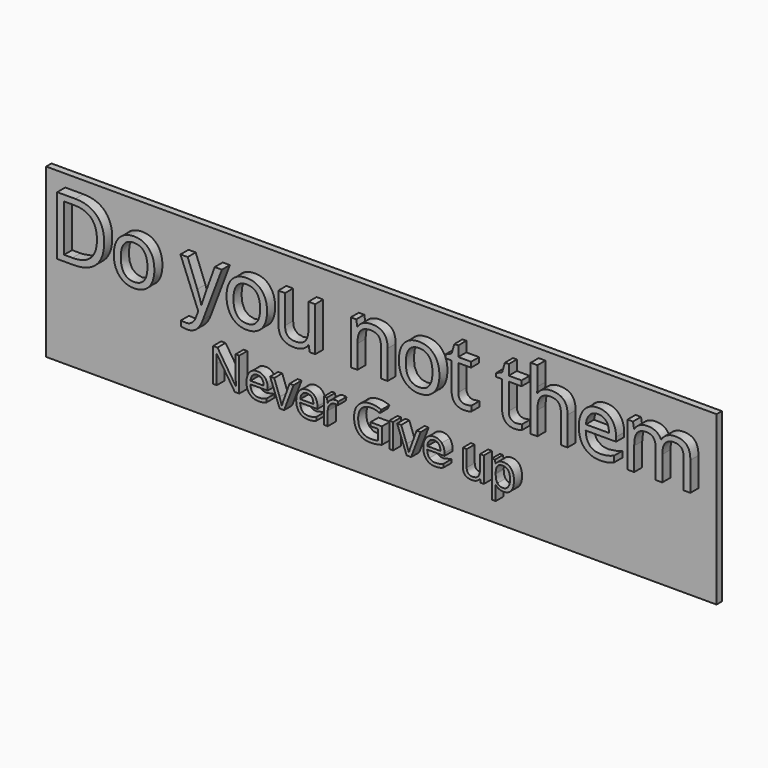
from build123d import *

# Parameters (mm, degrees)
F0_TEXT_SIZE = 62.4328592999
F1_DEPTH     = 12.7
F0_W         = 2.8789125633
F0_H         = 18.9986041025
F2_DEPTH     = 12.7
F3_DEPTH     = 5.08


# Not quite as in the source:
# - Text() gives the source's letters only with a copy of the font that has no kerning and outlines rounded to 1/6400 em; it was checked with that copy


with BuildPart() as f1:
    # F0 (on Front) → F1 (new body)
    with BuildSketch(Plane.XZ):
        with Locations((-245.5882579088, 73.1566213071)):
            Text('Do you not them', F0_TEXT_SIZE, font='Open Sans', text_align=(TextAlign.LEFT, TextAlign.BOTTOM))
    extrude(amount=F1_DEPTH)


with BuildPart() as f2:
    # F0 (on Front) → F2 (new body)
    with BuildSketch(Plane.XZ):
        with BuildLine():
            Line((-104.9163470416, 28.2049644738), (-101.5548421989, 28.2049644738))
            Line((-101.5548421989, 28.2049644738), (-101.5548421989, 53.5493796985))
            Line((-101.5548421989, 53.5493796985), (-104.3117199329, 53.5493796985))
            Line((-104.3117199329, 53.5493796985), (-104.3117199329, 39.0050468644))
            add(Edge.make_bspline(
                [(-104.2229673298, 35.3717371747), (-104.3450021591, 37.9122804386), (-104.3117199329, 39.0050468644)],
                knots=[0, 0, 0, 1, 1, 1], degree=2))
            add(Edge.make_bspline(
                [(-104.0676502744, 32.3652427445), (-104.1009325005, 32.8311939108), (-104.2229673298, 35.3717371747)],
                knots=[0, 0, 0, 1, 1, 1], degree=2))
            Line((-104.0676502744, 32.3652427445), (-104.2063262167, 32.3652427445))
            Line((-104.2063262167, 32.3652427445), (-118.0239971129, 53.5493796985))
            Line((-118.0239971129, 53.5493796985), (-121.3522197294, 53.5493796985))
            Line((-121.3522197294, 53.5493796985), (-121.3522197294, 28.2049644738))
            Line((-121.3522197294, 28.2049644738), (-118.6286242216, 28.2049644738))
            Line((-118.6286242216, 28.2049644738), (-118.6286242216, 42.6106213656))
            add(Edge.make_bspline(
                [(-118.9059761063, 49.4723069933), (-118.6286242216, 45.7280565497), (-118.6286242216, 42.6106213656)],
                knots=[0, 0, 0, 1, 1, 1], degree=2))
            Line((-118.9059761063, 49.4723069933), (-118.7673001639, 49.4723069933))
            Line((-118.7673001639, 49.4723069933), (-104.9163470416, 28.2049644738))
        make_face()
        with BuildLine():
            add(Edge.make_bspline(
                [(-86.9938682517, 27.8555010991), (-91.2040698616, 27.8555010991), (-93.6419929282, 30.4237795515)],
                knots=[0, 0, 0, 1, 1, 1], degree=2))
            add(Edge.make_bspline(
                [(-83.7100219368, 28.1439470592), (-85.0690461719, 27.8555010991), (-86.9938682517, 27.8555010991)],
                knots=[0, 0, 0, 1, 1, 1], degree=2))
            add(Edge.make_bspline(
                [(-80.8255623358, 29.0869434672), (-82.3509977017, 28.4323930193), (-83.7100219368, 28.1439470592)],
                knots=[0, 0, 0, 1, 1, 1], degree=2))
            Line((-80.8255623358, 29.0869434672), (-80.8255623358, 31.6552219196))
            add(Edge.make_bspline(
                [(-86.8884745355, 30.3738562123), (-83.8209626907, 30.3738562123), (-80.8255623358, 31.6552219196)],
                knots=[0, 0, 0, 1, 1, 1], degree=2))
            add(Edge.make_bspline(
                [(-91.4037632186, 32.1073054917), (-89.800669325, 30.3738562123), (-86.8884745355, 30.3738562123)],
                knots=[0, 0, 0, 1, 1, 1], degree=2))
            add(Edge.make_bspline(
                [(-93.0956097153, 37.1856185007), (-93.0068571122, 33.8407547711), (-91.4037632186, 32.1073054917)],
                knots=[0, 0, 0, 1, 1, 1], degree=2))
            Line((-93.0956097153, 37.1856185007), (-80.0101477948, 37.1856185007))
            Line((-80.0101477948, 37.1856185007), (-80.0101477948, 39.0050468644))
            add(Edge.make_bspline(
                [(-82.0902869301, 45.2038614876), (-80.0101477948, 42.8546910241), (-80.0101477948, 39.0050468644)],
                knots=[0, 0, 0, 1, 1, 1], degree=2))
            add(Edge.make_bspline(
                [(-87.7371713028, 47.5530319511), (-84.1704260654, 47.5530319511), (-82.0902869301, 45.2038614876)],
                knots=[0, 0, 0, 1, 1, 1], degree=2))
            add(Edge.make_bspline(
                [(-93.8167246156, 44.8488510752), (-91.5535332363, 47.5530319511), (-87.7371713028, 47.5530319511)],
                knots=[0, 0, 0, 1, 1, 1], degree=2))
            add(Edge.make_bspline(
                [(-96.0799159948, 37.5461759508), (-96.0799159948, 42.1446701993), (-93.8167246156, 44.8488510752)],
                knots=[0, 0, 0, 1, 1, 1], degree=2))
            add(Edge.make_bspline(
                [(-93.6419929282, 30.4237795515), (-96.0799159948, 32.9920580039), (-96.0799159948, 37.5461759508)],
                knots=[0, 0, 0, 1, 1, 1], degree=2))
        make_face()
        with BuildLine():
            add(Edge.make_bspline(
                [(-87.7760005666, 45.1400705541), (-90.0613800966, 45.1400705541), (-91.4231778505, 43.6506909332)],
                knots=[0, 0, 0, 1, 1, 1], degree=2))
            add(Edge.make_bspline(
                [(-84.3063284889, 43.6922937159), (-85.5183562251, 45.1400705541), (-87.7760005666, 45.1400705541)],
                knots=[0, 0, 0, 1, 1, 1], degree=2))
            add(Edge.make_bspline(
                [(-83.0943007527, 39.5264684076), (-83.0943007527, 42.2445168778), (-84.3063284889, 43.6922937159)],
                knots=[0, 0, 0, 1, 1, 1], degree=2))
            Line((-83.0943007527, 39.5264684076), (-93.029045263, 39.5264684076))
            add(Edge.make_bspline(
                [(-91.4231778505, 43.6506909332), (-92.7849756044, 42.1613113124), (-93.029045263, 39.5264684076)],
                knots=[0, 0, 0, 1, 1, 1], degree=2))
        make_face(mode=Mode.SUBTRACT)
        with BuildLine():
            Line((-78.1518901672, 47.2035685764), (-70.9407411648, 28.2049644738))
            Line((-70.9407411648, 28.2049644738), (-67.5792363222, 28.2049644738))
            Line((-67.5792363222, 28.2049644738), (-60.3680873198, 47.2035685764))
            Line((-60.3680873198, 47.2035685764), (-63.4522402777, 47.2035685764))
            add(Edge.make_bspline(
                [(-68.0008111869, 34.6090194918), (-66.9857032889, 37.4962526116), (-63.4522402777, 47.2035685764)],
                knots=[0, 0, 0, 1, 1, 1], degree=2))
            add(Edge.make_bspline(
                [(-69.2045183666, 30.8065251524), (-69.015919085, 31.7217863719), (-68.0008111869, 34.6090194918)],
                knots=[0, 0, 0, 1, 1, 1], degree=2))
            Line((-69.2045183666, 30.8065251524), (-69.3431943089, 30.8065251524))
            add(Edge.make_bspline(
                [(-70.974023391, 35.9375350195), (-69.5872639675, 31.9824971436), (-69.3431943089, 30.8065251524)],
                knots=[0, 0, 0, 1, 1, 1], degree=2))
            Line((-70.974023391, 35.9375350195), (-75.0677372093, 47.2035685764))
            Line((-75.0677372093, 47.2035685764), (-78.1518901672, 47.2035685764))
        make_face()
        with BuildLine():
            add(Edge.make_bspline(
                [(-49.2906530445, 27.8555010991), (-53.5008546544, 27.8555010991), (-55.938777721, 30.4237795515)],
                knots=[0, 0, 0, 1, 1, 1], degree=2))
            add(Edge.make_bspline(
                [(-46.0068067296, 28.1439470592), (-47.3658309646, 27.8555010991), (-49.2906530445, 27.8555010991)],
                knots=[0, 0, 0, 1, 1, 1], degree=2))
            add(Edge.make_bspline(
                [(-43.1223471286, 29.0869434672), (-44.6477824945, 28.4323930193), (-46.0068067296, 28.1439470592)],
                knots=[0, 0, 0, 1, 1, 1], degree=2))
            Line((-43.1223471286, 29.0869434672), (-43.1223471286, 31.6552219196))
            add(Edge.make_bspline(
                [(-49.1852593283, 30.3738562123), (-46.1177474834, 30.3738562123), (-43.1223471286, 31.6552219196)],
                knots=[0, 0, 0, 1, 1, 1], degree=2))
            add(Edge.make_bspline(
                [(-53.7005480114, 32.1073054917), (-52.0974541178, 30.3738562123), (-49.1852593283, 30.3738562123)],
                knots=[0, 0, 0, 1, 1, 1], degree=2))
            add(Edge.make_bspline(
                [(-55.3923945081, 37.1856185007), (-55.303641905, 33.8407547711), (-53.7005480114, 32.1073054917)],
                knots=[0, 0, 0, 1, 1, 1], degree=2))
            Line((-55.3923945081, 37.1856185007), (-42.3069325876, 37.1856185007))
            Line((-42.3069325876, 37.1856185007), (-42.3069325876, 39.0050468644))
            add(Edge.make_bspline(
                [(-44.3870717229, 45.2038614876), (-42.3069325876, 42.8546910241), (-42.3069325876, 39.0050468644)],
                knots=[0, 0, 0, 1, 1, 1], degree=2))
            add(Edge.make_bspline(
                [(-50.0339560955, 47.5530319511), (-46.4672108582, 47.5530319511), (-44.3870717229, 45.2038614876)],
                knots=[0, 0, 0, 1, 1, 1], degree=2))
            add(Edge.make_bspline(
                [(-56.1135094083, 44.8488510752), (-53.8503180291, 47.5530319511), (-50.0339560955, 47.5530319511)],
                knots=[0, 0, 0, 1, 1, 1], degree=2))
            add(Edge.make_bspline(
                [(-58.3767007875, 37.5461759508), (-58.3767007875, 42.1446701993), (-56.1135094083, 44.8488510752)],
                knots=[0, 0, 0, 1, 1, 1], degree=2))
            add(Edge.make_bspline(
                [(-55.938777721, 30.4237795515), (-58.3767007875, 32.9920580039), (-58.3767007875, 37.5461759508)],
                knots=[0, 0, 0, 1, 1, 1], degree=2))
        make_face()
        with BuildLine():
            add(Edge.make_bspline(
                [(-50.0727853594, 45.1400705541), (-52.3581648894, 45.1400705541), (-53.7199626433, 43.6506909332)],
                knots=[0, 0, 0, 1, 1, 1], degree=2))
            add(Edge.make_bspline(
                [(-46.6031132817, 43.6922937159), (-47.8151410179, 45.1400705541), (-50.0727853594, 45.1400705541)],
                knots=[0, 0, 0, 1, 1, 1], degree=2))
            add(Edge.make_bspline(
                [(-45.3910855455, 39.5264684076), (-45.3910855455, 42.2445168778), (-46.6031132817, 43.6922937159)],
                knots=[0, 0, 0, 1, 1, 1], degree=2))
            Line((-45.3910855455, 39.5264684076), (-55.3258300558, 39.5264684076))
            add(Edge.make_bspline(
                [(-53.7199626433, 43.6506909332), (-55.0817603972, 42.1613113124), (-55.3258300558, 39.5264684076)],
                knots=[0, 0, 0, 1, 1, 1], degree=2))
        make_face(mode=Mode.SUBTRACT)
        with BuildLine():
            add(Edge.make_bspline(
                [(-28.7277843122, 47.5530319511), (-27.463059718, 47.5530319511), (-26.4590458953, 47.3422445187)],
                knots=[0, 0, 0, 1, 1, 1], degree=2))
            add(Edge.make_bspline(
                [(-32.0060835895, 46.5462446096), (-30.5139304498, 47.5530319511), (-28.7277843122, 47.5530319511)],
                knots=[0, 0, 0, 1, 1, 1], degree=2))
            add(Edge.make_bspline(
                [(-34.5521738911, 43.6867466783), (-33.4982367292, 45.5394572681), (-32.0060835895, 46.5462446096)],
                knots=[0, 0, 0, 1, 1, 1], degree=2))
            Line((-34.5521738911, 43.6867466783), (-34.6908498335, 43.6867466783))
            Line((-34.6908498335, 43.6867466783), (-35.0236720951, 47.2035685764))
            Line((-35.0236720951, 47.2035685764), (-37.3978042282, 47.2035685764))
            Line((-37.3978042282, 47.2035685764), (-37.3978042282, 28.2049644738))
            Line((-37.3978042282, 28.2049644738), (-34.518891665, 28.2049644738))
            Line((-34.518891665, 28.2049644738), (-34.518891665, 38.4004197557))
            add(Edge.make_bspline(
                [(-32.8825155452, 43.0627049377), (-34.518891665, 41.1905797159), (-34.518891665, 38.4004197557)],
                knots=[0, 0, 0, 1, 1, 1], degree=2))
            add(Edge.make_bspline(
                [(-28.9385717446, 44.9348301594), (-31.2461394254, 44.9348301594), (-32.8825155452, 43.0627049377)],
                knots=[0, 0, 0, 1, 1, 1], degree=2))
            add(Edge.make_bspline(
                [(-26.8584326093, 44.6741193878), (-28.0344046005, 44.9348301594), (-28.9385717446, 44.9348301594)],
                knots=[0, 0, 0, 1, 1, 1], degree=2))
            Line((-26.8584326093, 44.6741193878), (-26.4590458953, 47.3422445187))
        make_face()
        with BuildLine():
            Line((6.5180931965, 41.4845727137), (-2.0964563426, 41.4845727137))
            Line((-2.0964563426, 41.4845727137), (-2.0964563426, 38.8497298089))
            Line((-2.0964563426, 38.8497298089), (3.5670691432, 38.8497298089))
            Line((3.5670691432, 38.8497298089), (3.5670691432, 31.0505948109))
            add(Edge.make_bspline(
                [(-1.580581837, 30.4404206646), (1.0542610677, 30.4404206646), (3.5670691432, 31.0505948109)],
                knots=[0, 0, 0, 1, 1, 1], degree=2))
            add(Edge.make_bspline(
                [(-8.9387273383, 33.0919046824), (-6.4342398194, 30.4404206646), (-1.580581837, 30.4404206646)],
                knots=[0, 0, 0, 1, 1, 1], degree=2))
            add(Edge.make_bspline(
                [(-11.4432148572, 40.8743985673), (-11.4432148572, 35.7433887002), (-8.9387273383, 33.0919046824)],
                knots=[0, 0, 0, 1, 1, 1], degree=2))
            add(Edge.make_bspline(
                [(-8.8416541787, 48.5209900287), (-11.4432148572, 45.7668858136), (-11.4432148572, 40.8743985673)],
                knots=[0, 0, 0, 1, 1, 1], degree=2))
            add(Edge.make_bspline(
                [(-1.6138640632, 51.2750942439), (-6.2400935001, 51.2750942439), (-8.8416541787, 48.5209900287)],
                knots=[0, 0, 0, 1, 1, 1], degree=2))
            add(Edge.make_bspline(
                [(4.9926578306, 49.821770368), (1.5590414979, 51.2750942439), (-1.6138640632, 51.2750942439)],
                knots=[0, 0, 0, 1, 1, 1], degree=2))
            Line((4.9926578306, 49.821770368), (6.1353475956, 52.4233310466))
            add(Edge.make_bspline(
                [(-1.4252647816, 53.9099371486), (2.6351668106, 53.9099371486), (6.1353475956, 52.4233310466)],
                knots=[0, 0, 0, 1, 1, 1], degree=2))
            add(Edge.make_bspline(
                [(-8.4062117197, 52.342899), (-5.4246789591, 53.9099371486), (-1.4252647816, 53.9099371486)],
                knots=[0, 0, 0, 1, 1, 1], degree=2))
            add(Edge.make_bspline(
                [(-12.9741972608, 47.8026486473), (-11.3877444803, 50.7758608514), (-8.4062117197, 52.342899)],
                knots=[0, 0, 0, 1, 1, 1], degree=2))
            add(Edge.make_bspline(
                [(-14.5606500414, 40.8743985673), (-14.5606500414, 44.8294364433), (-12.9741972608, 47.8026486473)],
                knots=[0, 0, 0, 1, 1, 1], degree=2))
            add(Edge.make_bspline(
                [(-11.3544622541, 31.2807968753), (-14.5606500414, 34.7060926514), (-14.5606500414, 40.8743985673)],
                knots=[0, 0, 0, 1, 1, 1], degree=2))
            add(Edge.make_bspline(
                [(-2.3959963781, 27.8555010991), (-8.1482744669, 27.8555010991), (-11.3544622541, 31.2807968753)],
                knots=[0, 0, 0, 1, 1, 1], degree=2))
            add(Edge.make_bspline(
                [(2.4243793782, 28.1855498419), (0.3442402429, 27.8555010991), (-2.3959963781, 27.8555010991)],
                knots=[0, 0, 0, 1, 1, 1], degree=2))
            add(Edge.make_bspline(
                [(6.5180931965, 29.1590549572), (4.5045185135, 28.5155985847), (2.4243793782, 28.1855498419)],
                knots=[0, 0, 0, 1, 1, 1], degree=2))
            Line((6.5180931965, 29.1590549572), (6.5180931965, 41.4845727137))
        make_face()
        with Locations((13.6044338508, 37.7042665251)):
            Rectangle(F0_W, F0_H)
        with BuildLine():
            Line((18.0947608642, 47.2035685764), (25.3059098666, 28.2049644738))
            Line((25.3059098666, 28.2049644738), (28.6674147093, 28.2049644738))
            Line((28.6674147093, 28.2049644738), (35.8785637117, 47.2035685764))
            Line((35.8785637117, 47.2035685764), (32.7944107537, 47.2035685764))
            add(Edge.make_bspline(
                [(28.2458398445, 34.6090194918), (29.2609477425, 37.4962526116), (32.7944107537, 47.2035685764)],
                knots=[0, 0, 0, 1, 1, 1], degree=2))
            add(Edge.make_bspline(
                [(27.0421326649, 30.8065251524), (27.2307319465, 31.7217863719), (28.2458398445, 34.6090194918)],
                knots=[0, 0, 0, 1, 1, 1], degree=2))
            Line((27.0421326649, 30.8065251524), (26.9034567225, 30.8065251524))
            add(Edge.make_bspline(
                [(25.2726276404, 35.9375350195), (26.659387064, 31.9824971436), (26.9034567225, 30.8065251524)],
                knots=[0, 0, 0, 1, 1, 1], degree=2))
            Line((25.2726276404, 35.9375350195), (21.1789138221, 47.2035685764))
            Line((21.1789138221, 47.2035685764), (18.0947608642, 47.2035685764))
        make_face()
        with BuildLine():
            add(Edge.make_bspline(
                [(46.9559979869, 27.8555010991), (42.745796377, 27.8555010991), (40.3078733105, 30.4237795515)],
                knots=[0, 0, 0, 1, 1, 1], degree=2))
            add(Edge.make_bspline(
                [(50.2398443019, 28.1439470592), (48.8808200668, 27.8555010991), (46.9559979869, 27.8555010991)],
                knots=[0, 0, 0, 1, 1, 1], degree=2))
            add(Edge.make_bspline(
                [(53.1243039028, 29.0869434672), (51.5988685369, 28.4323930193), (50.2398443019, 28.1439470592)],
                knots=[0, 0, 0, 1, 1, 1], degree=2))
            Line((53.1243039028, 29.0869434672), (53.1243039028, 31.6552219196))
            add(Edge.make_bspline(
                [(47.0613917031, 30.3738562123), (50.128903548, 30.3738562123), (53.1243039028, 31.6552219196)],
                knots=[0, 0, 0, 1, 1, 1], degree=2))
            add(Edge.make_bspline(
                [(42.5461030201, 32.1073054917), (44.1491969137, 30.3738562123), (47.0613917031, 30.3738562123)],
                knots=[0, 0, 0, 1, 1, 1], degree=2))
            add(Edge.make_bspline(
                [(40.8542565233, 37.1856185007), (40.9430091264, 33.8407547711), (42.5461030201, 32.1073054917)],
                knots=[0, 0, 0, 1, 1, 1], degree=2))
            Line((40.8542565233, 37.1856185007), (53.9397184439, 37.1856185007))
            Line((53.9397184439, 37.1856185007), (53.9397184439, 39.0050468644))
            add(Edge.make_bspline(
                [(51.8595793086, 45.2038614876), (53.9397184439, 42.8546910241), (53.9397184439, 39.0050468644)],
                knots=[0, 0, 0, 1, 1, 1], degree=2))
            add(Edge.make_bspline(
                [(46.2126949359, 47.5530319511), (49.7794401732, 47.5530319511), (51.8595793086, 45.2038614876)],
                knots=[0, 0, 0, 1, 1, 1], degree=2))
            add(Edge.make_bspline(
                [(40.1331416231, 44.8488510752), (42.3963330023, 47.5530319511), (46.2126949359, 47.5530319511)],
                knots=[0, 0, 0, 1, 1, 1], degree=2))
            add(Edge.make_bspline(
                [(37.8699502439, 37.5461759508), (37.8699502439, 42.1446701993), (40.1331416231, 44.8488510752)],
                knots=[0, 0, 0, 1, 1, 1], degree=2))
            add(Edge.make_bspline(
                [(40.3078733105, 30.4237795515), (37.8699502439, 32.9920580039), (37.8699502439, 37.5461759508)],
                knots=[0, 0, 0, 1, 1, 1], degree=2))
        make_face()
        with BuildLine():
            add(Edge.make_bspline(
                [(46.173865672, 45.1400705541), (43.888486142, 45.1400705541), (42.5266883881, 43.6506909332)],
                knots=[0, 0, 0, 1, 1, 1], degree=2))
            add(Edge.make_bspline(
                [(49.6435377497, 43.6922937159), (48.4315100136, 45.1400705541), (46.173865672, 45.1400705541)],
                knots=[0, 0, 0, 1, 1, 1], degree=2))
            add(Edge.make_bspline(
                [(50.8555654859, 39.5264684076), (50.8555654859, 42.2445168778), (49.6435377497, 43.6922937159)],
                knots=[0, 0, 0, 1, 1, 1], degree=2))
            Line((50.8555654859, 39.5264684076), (40.9208209757, 39.5264684076))
            add(Edge.make_bspline(
                [(42.5266883881, 43.6506909332), (41.1648906342, 42.1613113124), (40.9208209757, 39.5264684076)],
                knots=[0, 0, 0, 1, 1, 1], degree=2))
        make_face(mode=Mode.SUBTRACT)
        with BuildLine():
            Line((70.7805248834, 34.8780508199), (70.7805248834, 47.2035685764))
            Line((70.7805248834, 47.2035685764), (67.8683300939, 47.2035685764))
            Line((67.8683300939, 47.2035685764), (67.8683300939, 34.7726571037))
            add(Edge.make_bspline(
                [(69.590685298, 29.5029712943), (67.8683300939, 31.1504414894), (67.8683300939, 34.7726571037)],
                knots=[0, 0, 0, 1, 1, 1], degree=2))
            add(Edge.make_bspline(
                [(74.7799390608, 27.8555010991), (71.313040502, 27.8555010991), (69.590685298, 29.5029712943)],
                knots=[0, 0, 0, 1, 1, 1], degree=2))
            add(Edge.make_bspline(
                [(78.3633254113, 28.601577669), (76.7935137438, 27.8555010991), (74.7799390608, 27.8555010991)],
                knots=[0, 0, 0, 1, 1, 1], degree=2))
            add(Edge.make_bspline(
                [(80.8151160721, 30.7510547755), (79.9331370787, 29.3476542388), (78.3633254113, 28.601577669)],
                knots=[0, 0, 0, 1, 1, 1], degree=2))
            Line((80.8151160721, 30.7510547755), (80.9704331275, 30.7510547755))
            Line((80.9704331275, 30.7510547755), (81.3864609546, 28.2049644738))
            Line((81.3864609546, 28.2049644738), (83.7605930877, 28.2049644738))
            Line((83.7605930877, 28.2049644738), (83.7605930877, 47.2035685764))
            Line((83.7605930877, 47.2035685764), (80.8816805244, 47.2035685764))
            Line((80.8816805244, 47.2035685764), (80.8816805244, 37.2189007269))
            add(Edge.make_bspline(
                [(79.5060151763, 31.8965180593), (80.8816805244, 33.5245736225), (80.8816805244, 37.2189007269)],
                knots=[0, 0, 0, 1, 1, 1], degree=2))
            add(Edge.make_bspline(
                [(75.1460435487, 30.2684624961), (78.1303498281, 30.2684624961), (79.5060151763, 31.8965180593)],
                knots=[0, 0, 0, 1, 1, 1], degree=2))
            add(Edge.make_bspline(
                [(71.8372355641, 31.4111522611), (72.8939462448, 30.2684624961), (75.1460435487, 30.2684624961)],
                knots=[0, 0, 0, 1, 1, 1], degree=2))
            add(Edge.make_bspline(
                [(70.7805248834, 34.8780508199), (70.7805248834, 32.5538420261), (71.8372355641, 31.4111522611)],
                knots=[0, 0, 0, 1, 1, 1], degree=2))
        make_face()
        with BuildLine():
            add(Edge.make_bspline(
                [(98.7043126358, 27.8555010991), (96.8460550082, 27.8555010991), (95.3122990858, 28.5405602543)],
                knots=[0, 0, 0, 1, 1, 1], degree=2))
            add(Edge.make_bspline(
                [(104.503740545, 30.4487412211), (102.4152808532, 27.8555010991), (98.7043126358, 27.8555010991)],
                knots=[0, 0, 0, 1, 1, 1], degree=2))
            add(Edge.make_bspline(
                [(106.5922002369, 37.723681157), (106.5922002369, 33.0419813432), (104.503740545, 30.4487412211)],
                knots=[0, 0, 0, 1, 1, 1], degree=2))
            add(Edge.make_bspline(
                [(104.5370227712, 44.9681123856), (106.5922002369, 42.3831928201), (106.5922002369, 37.723681157)],
                knots=[0, 0, 0, 1, 1, 1], degree=2))
            add(Edge.make_bspline(
                [(98.7043126358, 47.5530319511), (102.4818453055, 47.5530319511), (104.5370227712, 44.9681123856)],
                knots=[0, 0, 0, 1, 1, 1], degree=2))
            add(Edge.make_bspline(
                [(95.3233931612, 46.8596522393), (96.796131669, 47.5530319511), (98.7043126358, 47.5530319511)],
                knots=[0, 0, 0, 1, 1, 1], degree=2))
            add(Edge.make_bspline(
                [(92.7412471145, 44.6020078978), (93.8506546534, 46.1662725275), (95.3233931612, 46.8596522393)],
                knots=[0, 0, 0, 1, 1, 1], degree=2))
            Line((92.7412471145, 44.6020078978), (92.6025711722, 44.6020078978))
            Line((92.6025711722, 44.6020078978), (92.2031844582, 47.2035685764))
            Line((92.2031844582, 47.2035685764), (89.8623345513, 47.2035685764))
            Line((89.8623345513, 47.2035685764), (89.8623345513, 19.6736205002))
            Line((89.8623345513, 19.6736205002), (92.7412471145, 19.6736205002))
            Line((92.7412471145, 19.6736205002), (92.7412471145, 27.494943649))
            add(Edge.make_bspline(
                [(92.5304596822, 30.651208097), (92.7412471145, 28.9870967887), (92.7412471145, 27.494943649)],
                knots=[0, 0, 0, 1, 1, 1], degree=2))
            Line((92.5304596822, 30.651208097), (92.7412471145, 30.651208097))
            add(Edge.make_bspline(
                [(95.3122990858, 28.5405602543), (93.7785431634, 29.2256194096), (92.7412471145, 30.651208097)],
                knots=[0, 0, 0, 1, 1, 1], degree=2))
        make_face()
        with BuildLine():
            add(Edge.make_bspline(
                [(98.2882848087, 45.106788328), (95.3760900193, 45.106788328), (94.07530968, 43.4953738778)],
                knots=[0, 0, 0, 1, 1, 1], degree=2))
            add(Edge.make_bspline(
                [(102.2128139773, 43.2097014366), (100.8177339972, 45.106788328), (98.2882848087, 45.106788328)],
                knots=[0, 0, 0, 1, 1, 1], degree=2))
            add(Edge.make_bspline(
                [(103.6078939574, 37.7569633832), (103.6078939574, 41.3126145452), (102.2128139773, 43.2097014366)],
                knots=[0, 0, 0, 1, 1, 1], degree=2))
            add(Edge.make_bspline(
                [(102.2128139773, 32.2626225471), (103.6078939574, 34.2567825982), (103.6078939574, 37.7569633832)],
                knots=[0, 0, 0, 1, 1, 1], degree=2))
            add(Edge.make_bspline(
                [(98.354849261, 30.2684624961), (100.8177339972, 30.2684624961), (102.2128139773, 32.2626225471)],
                knots=[0, 0, 0, 1, 1, 1], degree=2))
            add(Edge.make_bspline(
                [(94.07530968, 31.993591219), (95.4093722454, 30.2684624961), (98.354849261, 30.2684624961)],
                knots=[0, 0, 0, 1, 1, 1], degree=2))
            add(Edge.make_bspline(
                [(92.7412471145, 37.723681157), (92.7412471145, 33.7187199418), (94.07530968, 31.993591219)],
                knots=[0, 0, 0, 1, 1, 1], degree=2))
            Line((92.7412471145, 37.723681157), (92.7412471145, 38.3615904919))
            add(Edge.make_bspline(
                [(94.07530968, 43.4953738778), (92.7745293407, 41.8839594277), (92.7412471145, 38.3615904919)],
                knots=[0, 0, 0, 1, 1, 1], degree=2))
        make_face(mode=Mode.SUBTRACT)
    extrude(amount=F2_DEPTH)


with BuildPart() as f3:
    # F0 (on Front) → F3 (new body)
    with BuildSketch(Plane.XZ):
        Polygon((-254, 0), (0, 0), (254, 0), (254, 127), (-254, 127), align=None)
        with BuildLine():
            add(Edge.make_bspline(
                [(-83.7100219368, 28.1439470592), (-85.0690461719, 27.8555010991), (-86.9938682517, 27.8555010991)],
                knots=[0, 0, 0, 1, 1, 1], degree=2))
            add(Edge.make_bspline(
                [(-86.9938682517, 27.8555010991), (-91.2040698616, 27.8555010991), (-93.6419929282, 30.4237795515)],
                knots=[0, 0, 0, 1, 1, 1], degree=2))
            add(Edge.make_bspline(
                [(-93.6419929282, 30.4237795515), (-96.0799159948, 32.9920580039), (-96.0799159948, 37.5461759508)],
                knots=[0, 0, 0, 1, 1, 1], degree=2))
            add(Edge.make_bspline(
                [(-96.0799159948, 37.5461759508), (-96.0799159948, 42.1446701993), (-93.8167246156, 44.8488510752)],
                knots=[0, 0, 0, 1, 1, 1], degree=2))
            add(Edge.make_bspline(
                [(-93.8167246156, 44.8488510752), (-91.5535332363, 47.5530319511), (-87.7371713028, 47.5530319511)],
                knots=[0, 0, 0, 1, 1, 1], degree=2))
            add(Edge.make_bspline(
                [(-87.7371713028, 47.5530319511), (-84.1704260654, 47.5530319511), (-82.0902869301, 45.2038614876)],
                knots=[0, 0, 0, 1, 1, 1], degree=2))
            add(Edge.make_bspline(
                [(-82.0902869301, 45.2038614876), (-80.0101477948, 42.8546910241), (-80.0101477948, 39.0050468644)],
                knots=[0, 0, 0, 1, 1, 1], degree=2))
            Line((-80.0101477948, 39.0050468644), (-80.0101477948, 37.1856185007))
            Line((-80.0101477948, 37.1856185007), (-93.0956097153, 37.1856185007))
            add(Edge.make_bspline(
                [(-93.0956097153, 37.1856185007), (-93.0068571122, 33.8407547711), (-91.4037632186, 32.1073054917)],
                knots=[0, 0, 0, 1, 1, 1], degree=2))
            add(Edge.make_bspline(
                [(-91.4037632186, 32.1073054917), (-89.800669325, 30.3738562123), (-86.8884745355, 30.3738562123)],
                knots=[0, 0, 0, 1, 1, 1], degree=2))
            add(Edge.make_bspline(
                [(-86.8884745355, 30.3738562123), (-83.8209626907, 30.3738562123), (-80.8255623358, 31.6552219196)],
                knots=[0, 0, 0, 1, 1, 1], degree=2))
            Line((-80.8255623358, 31.6552219196), (-80.8255623358, 29.0869434672))
            add(Edge.make_bspline(
                [(-80.8255623358, 29.0869434672), (-82.3509977017, 28.4323930193), (-83.7100219368, 28.1439470592)],
                knots=[0, 0, 0, 1, 1, 1], degree=2))
        make_face(mode=Mode.SUBTRACT)
        with BuildLine():
            Line((-67.5792363222, 28.2049644738), (-70.9407411648, 28.2049644738))
            Line((-70.9407411648, 28.2049644738), (-78.1518901672, 47.2035685764))
            Line((-78.1518901672, 47.2035685764), (-75.0677372093, 47.2035685764))
            Line((-75.0677372093, 47.2035685764), (-70.974023391, 35.9375350195))
            add(Edge.make_bspline(
                [(-70.974023391, 35.9375350195), (-69.5872639675, 31.9824971436), (-69.3431943089, 30.8065251524)],
                knots=[0, 0, 0, 1, 1, 1], degree=2))
            Line((-69.3431943089, 30.8065251524), (-69.2045183666, 30.8065251524))
            add(Edge.make_bspline(
                [(-69.2045183666, 30.8065251524), (-69.015919085, 31.7217863719), (-68.0008111869, 34.6090194918)],
                knots=[0, 0, 0, 1, 1, 1], degree=2))
            add(Edge.make_bspline(
                [(-68.0008111869, 34.6090194918), (-66.9857032889, 37.4962526116), (-63.4522402777, 47.2035685764)],
                knots=[0, 0, 0, 1, 1, 1], degree=2))
            Line((-63.4522402777, 47.2035685764), (-60.3680873198, 47.2035685764))
            Line((-60.3680873198, 47.2035685764), (-67.5792363222, 28.2049644738))
        make_face(mode=Mode.SUBTRACT)
        with BuildLine():
            Line((-101.5548421989, 53.5493796985), (-101.5548421989, 28.2049644738))
            Line((-101.5548421989, 28.2049644738), (-104.9163470416, 28.2049644738))
            Line((-104.9163470416, 28.2049644738), (-118.7673001639, 49.4723069933))
            Line((-118.7673001639, 49.4723069933), (-118.9059761063, 49.4723069933))
            add(Edge.make_bspline(
                [(-118.9059761063, 49.4723069933), (-118.6286242216, 45.7280565497), (-118.6286242216, 42.6106213656)],
                knots=[0, 0, 0, 1, 1, 1], degree=2))
            Line((-118.6286242216, 42.6106213656), (-118.6286242216, 28.2049644738))
            Line((-118.6286242216, 28.2049644738), (-121.3522197294, 28.2049644738))
            Line((-121.3522197294, 28.2049644738), (-121.3522197294, 53.5493796985))
            Line((-121.3522197294, 53.5493796985), (-118.0239971129, 53.5493796985))
            Line((-118.0239971129, 53.5493796985), (-104.2063262167, 32.3652427445))
            Line((-104.2063262167, 32.3652427445), (-104.0676502744, 32.3652427445))
            add(Edge.make_bspline(
                [(-104.0676502744, 32.3652427445), (-104.1009325005, 32.8311939108), (-104.2229673298, 35.3717371747)],
                knots=[0, 0, 0, 1, 1, 1], degree=2))
            add(Edge.make_bspline(
                [(-104.2229673298, 35.3717371747), (-104.3450021591, 37.9122804386), (-104.3117199329, 39.0050468644)],
                knots=[0, 0, 0, 1, 1, 1], degree=2))
            Line((-104.3117199329, 39.0050468644), (-104.3117199329, 53.5493796985))
            Line((-104.3117199329, 53.5493796985), (-101.5548421989, 53.5493796985))
        make_face(mode=Mode.SUBTRACT)
        with BuildLine():
            add(Edge.make_bspline(
                [(-46.0068067296, 28.1439470592), (-47.3658309646, 27.8555010991), (-49.2906530445, 27.8555010991)],
                knots=[0, 0, 0, 1, 1, 1], degree=2))
            add(Edge.make_bspline(
                [(-49.2906530445, 27.8555010991), (-53.5008546544, 27.8555010991), (-55.938777721, 30.4237795515)],
                knots=[0, 0, 0, 1, 1, 1], degree=2))
            add(Edge.make_bspline(
                [(-55.938777721, 30.4237795515), (-58.3767007875, 32.9920580039), (-58.3767007875, 37.5461759508)],
                knots=[0, 0, 0, 1, 1, 1], degree=2))
            add(Edge.make_bspline(
                [(-58.3767007875, 37.5461759508), (-58.3767007875, 42.1446701993), (-56.1135094083, 44.8488510752)],
                knots=[0, 0, 0, 1, 1, 1], degree=2))
            add(Edge.make_bspline(
                [(-56.1135094083, 44.8488510752), (-53.8503180291, 47.5530319511), (-50.0339560955, 47.5530319511)],
                knots=[0, 0, 0, 1, 1, 1], degree=2))
            add(Edge.make_bspline(
                [(-50.0339560955, 47.5530319511), (-46.4672108582, 47.5530319511), (-44.3870717229, 45.2038614876)],
                knots=[0, 0, 0, 1, 1, 1], degree=2))
            add(Edge.make_bspline(
                [(-44.3870717229, 45.2038614876), (-42.3069325876, 42.8546910241), (-42.3069325876, 39.0050468644)],
                knots=[0, 0, 0, 1, 1, 1], degree=2))
            Line((-42.3069325876, 39.0050468644), (-42.3069325876, 37.1856185007))
            Line((-42.3069325876, 37.1856185007), (-55.3923945081, 37.1856185007))
            add(Edge.make_bspline(
                [(-55.3923945081, 37.1856185007), (-55.303641905, 33.8407547711), (-53.7005480114, 32.1073054917)],
                knots=[0, 0, 0, 1, 1, 1], degree=2))
            add(Edge.make_bspline(
                [(-53.7005480114, 32.1073054917), (-52.0974541178, 30.3738562123), (-49.1852593283, 30.3738562123)],
                knots=[0, 0, 0, 1, 1, 1], degree=2))
            add(Edge.make_bspline(
                [(-49.1852593283, 30.3738562123), (-46.1177474834, 30.3738562123), (-43.1223471286, 31.6552219196)],
                knots=[0, 0, 0, 1, 1, 1], degree=2))
            Line((-43.1223471286, 31.6552219196), (-43.1223471286, 29.0869434672))
            add(Edge.make_bspline(
                [(-43.1223471286, 29.0869434672), (-44.6477824945, 28.4323930193), (-46.0068067296, 28.1439470592)],
                knots=[0, 0, 0, 1, 1, 1], degree=2))
        make_face(mode=Mode.SUBTRACT)
        with BuildLine():
            add(Edge.make_bspline(
                [(-32.0060835895, 46.5462446096), (-30.5139304498, 47.5530319511), (-28.7277843122, 47.5530319511)],
                knots=[0, 0, 0, 1, 1, 1], degree=2))
            add(Edge.make_bspline(
                [(-28.7277843122, 47.5530319511), (-27.463059718, 47.5530319511), (-26.4590458953, 47.3422445187)],
                knots=[0, 0, 0, 1, 1, 1], degree=2))
            Line((-26.4590458953, 47.3422445187), (-26.8584326093, 44.6741193878))
            add(Edge.make_bspline(
                [(-26.8584326093, 44.6741193878), (-28.0344046005, 44.9348301594), (-28.9385717446, 44.9348301594)],
                knots=[0, 0, 0, 1, 1, 1], degree=2))
            add(Edge.make_bspline(
                [(-28.9385717446, 44.9348301594), (-31.2461394254, 44.9348301594), (-32.8825155452, 43.0627049377)],
                knots=[0, 0, 0, 1, 1, 1], degree=2))
            add(Edge.make_bspline(
                [(-32.8825155452, 43.0627049377), (-34.518891665, 41.1905797159), (-34.518891665, 38.4004197557)],
                knots=[0, 0, 0, 1, 1, 1], degree=2))
            Line((-34.518891665, 38.4004197557), (-34.518891665, 28.2049644738))
            Line((-34.518891665, 28.2049644738), (-37.3978042282, 28.2049644738))
            Line((-37.3978042282, 28.2049644738), (-37.3978042282, 47.2035685764))
            Line((-37.3978042282, 47.2035685764), (-35.0236720951, 47.2035685764))
            Line((-35.0236720951, 47.2035685764), (-34.6908498335, 43.6867466783))
            Line((-34.6908498335, 43.6867466783), (-34.5521738911, 43.6867466783))
            add(Edge.make_bspline(
                [(-34.5521738911, 43.6867466783), (-33.4982367292, 45.5394572681), (-32.0060835895, 46.5462446096)],
                knots=[0, 0, 0, 1, 1, 1], degree=2))
        make_face(mode=Mode.SUBTRACT)
        with BuildLine():
            Line((-2.0964563426, 38.8497298089), (-2.0964563426, 41.4845727137))
            Line((-2.0964563426, 41.4845727137), (6.5180931965, 41.4845727137))
            Line((6.5180931965, 41.4845727137), (6.5180931965, 29.1590549572))
            add(Edge.make_bspline(
                [(6.5180931965, 29.1590549572), (4.5045185135, 28.5155985847), (2.4243793782, 28.1855498419)],
                knots=[0, 0, 0, 1, 1, 1], degree=2))
            add(Edge.make_bspline(
                [(2.4243793782, 28.1855498419), (0.3442402429, 27.8555010991), (-2.3959963781, 27.8555010991)],
                knots=[0, 0, 0, 1, 1, 1], degree=2))
            add(Edge.make_bspline(
                [(-2.3959963781, 27.8555010991), (-8.1482744669, 27.8555010991), (-11.3544622541, 31.2807968753)],
                knots=[0, 0, 0, 1, 1, 1], degree=2))
            add(Edge.make_bspline(
                [(-11.3544622541, 31.2807968753), (-14.5606500414, 34.7060926514), (-14.5606500414, 40.8743985673)],
                knots=[0, 0, 0, 1, 1, 1], degree=2))
            add(Edge.make_bspline(
                [(-14.5606500414, 40.8743985673), (-14.5606500414, 44.8294364433), (-12.9741972608, 47.8026486473)],
                knots=[0, 0, 0, 1, 1, 1], degree=2))
            add(Edge.make_bspline(
                [(-12.9741972608, 47.8026486473), (-11.3877444803, 50.7758608514), (-8.4062117197, 52.342899)],
                knots=[0, 0, 0, 1, 1, 1], degree=2))
            add(Edge.make_bspline(
                [(-8.4062117197, 52.342899), (-5.4246789591, 53.9099371486), (-1.4252647816, 53.9099371486)],
                knots=[0, 0, 0, 1, 1, 1], degree=2))
            add(Edge.make_bspline(
                [(-1.4252647816, 53.9099371486), (2.6351668106, 53.9099371486), (6.1353475956, 52.4233310466)],
                knots=[0, 0, 0, 1, 1, 1], degree=2))
            Line((6.1353475956, 52.4233310466), (4.9926578306, 49.821770368))
            add(Edge.make_bspline(
                [(4.9926578306, 49.821770368), (1.5590414979, 51.2750942439), (-1.6138640632, 51.2750942439)],
                knots=[0, 0, 0, 1, 1, 1], degree=2))
            add(Edge.make_bspline(
                [(-1.6138640632, 51.2750942439), (-6.2400935001, 51.2750942439), (-8.8416541787, 48.5209900287)],
                knots=[0, 0, 0, 1, 1, 1], degree=2))
            add(Edge.make_bspline(
                [(-8.8416541787, 48.5209900287), (-11.4432148572, 45.7668858136), (-11.4432148572, 40.8743985673)],
                knots=[0, 0, 0, 1, 1, 1], degree=2))
            add(Edge.make_bspline(
                [(-11.4432148572, 40.8743985673), (-11.4432148572, 35.7433887002), (-8.9387273383, 33.0919046824)],
                knots=[0, 0, 0, 1, 1, 1], degree=2))
            add(Edge.make_bspline(
                [(-8.9387273383, 33.0919046824), (-6.4342398194, 30.4404206646), (-1.580581837, 30.4404206646)],
                knots=[0, 0, 0, 1, 1, 1], degree=2))
            add(Edge.make_bspline(
                [(-1.580581837, 30.4404206646), (1.0542610677, 30.4404206646), (3.5670691432, 31.0505948109)],
                knots=[0, 0, 0, 1, 1, 1], degree=2))
            Line((3.5670691432, 31.0505948109), (3.5670691432, 38.8497298089))
            Line((3.5670691432, 38.8497298089), (-2.0964563426, 38.8497298089))
        make_face(mode=Mode.SUBTRACT)
        with Locations((13.6044338508, 37.7042665251)):
            Rectangle(F0_W, F0_H, mode=Mode.SUBTRACT)
        with BuildLine():
            Line((28.6674147093, 28.2049644738), (25.3059098666, 28.2049644738))
            Line((25.3059098666, 28.2049644738), (18.0947608642, 47.2035685764))
            Line((18.0947608642, 47.2035685764), (21.1789138221, 47.2035685764))
            Line((21.1789138221, 47.2035685764), (25.2726276404, 35.9375350195))
            add(Edge.make_bspline(
                [(25.2726276404, 35.9375350195), (26.659387064, 31.9824971436), (26.9034567225, 30.8065251524)],
                knots=[0, 0, 0, 1, 1, 1], degree=2))
            Line((26.9034567225, 30.8065251524), (27.0421326649, 30.8065251524))
            add(Edge.make_bspline(
                [(27.0421326649, 30.8065251524), (27.2307319465, 31.7217863719), (28.2458398445, 34.6090194918)],
                knots=[0, 0, 0, 1, 1, 1], degree=2))
            add(Edge.make_bspline(
                [(28.2458398445, 34.6090194918), (29.2609477425, 37.4962526116), (32.7944107537, 47.2035685764)],
                knots=[0, 0, 0, 1, 1, 1], degree=2))
            Line((32.7944107537, 47.2035685764), (35.8785637117, 47.2035685764))
            Line((35.8785637117, 47.2035685764), (28.6674147093, 28.2049644738))
        make_face(mode=Mode.SUBTRACT)
        with BuildLine():
            add(Edge.make_bspline(
                [(50.2398443019, 28.1439470592), (48.8808200668, 27.8555010991), (46.9559979869, 27.8555010991)],
                knots=[0, 0, 0, 1, 1, 1], degree=2))
            add(Edge.make_bspline(
                [(46.9559979869, 27.8555010991), (42.745796377, 27.8555010991), (40.3078733105, 30.4237795515)],
                knots=[0, 0, 0, 1, 1, 1], degree=2))
            add(Edge.make_bspline(
                [(40.3078733105, 30.4237795515), (37.8699502439, 32.9920580039), (37.8699502439, 37.5461759508)],
                knots=[0, 0, 0, 1, 1, 1], degree=2))
            add(Edge.make_bspline(
                [(37.8699502439, 37.5461759508), (37.8699502439, 42.1446701993), (40.1331416231, 44.8488510752)],
                knots=[0, 0, 0, 1, 1, 1], degree=2))
            add(Edge.make_bspline(
                [(40.1331416231, 44.8488510752), (42.3963330023, 47.5530319511), (46.2126949359, 47.5530319511)],
                knots=[0, 0, 0, 1, 1, 1], degree=2))
            add(Edge.make_bspline(
                [(46.2126949359, 47.5530319511), (49.7794401732, 47.5530319511), (51.8595793086, 45.2038614876)],
                knots=[0, 0, 0, 1, 1, 1], degree=2))
            add(Edge.make_bspline(
                [(51.8595793086, 45.2038614876), (53.9397184439, 42.8546910241), (53.9397184439, 39.0050468644)],
                knots=[0, 0, 0, 1, 1, 1], degree=2))
            Line((53.9397184439, 39.0050468644), (53.9397184439, 37.1856185007))
            Line((53.9397184439, 37.1856185007), (40.8542565233, 37.1856185007))
            add(Edge.make_bspline(
                [(40.8542565233, 37.1856185007), (40.9430091264, 33.8407547711), (42.5461030201, 32.1073054917)],
                knots=[0, 0, 0, 1, 1, 1], degree=2))
            add(Edge.make_bspline(
                [(42.5461030201, 32.1073054917), (44.1491969137, 30.3738562123), (47.0613917031, 30.3738562123)],
                knots=[0, 0, 0, 1, 1, 1], degree=2))
            add(Edge.make_bspline(
                [(47.0613917031, 30.3738562123), (50.128903548, 30.3738562123), (53.1243039028, 31.6552219196)],
                knots=[0, 0, 0, 1, 1, 1], degree=2))
            Line((53.1243039028, 31.6552219196), (53.1243039028, 29.0869434672))
            add(Edge.make_bspline(
                [(53.1243039028, 29.0869434672), (51.5988685369, 28.4323930193), (50.2398443019, 28.1439470592)],
                knots=[0, 0, 0, 1, 1, 1], degree=2))
        make_face(mode=Mode.SUBTRACT)
        with BuildLine():
            Line((67.8683300939, 47.2035685764), (70.7805248834, 47.2035685764))
            Line((70.7805248834, 47.2035685764), (70.7805248834, 34.8780508199))
            add(Edge.make_bspline(
                [(70.7805248834, 34.8780508199), (70.7805248834, 32.5538420261), (71.8372355641, 31.4111522611)],
                knots=[0, 0, 0, 1, 1, 1], degree=2))
            add(Edge.make_bspline(
                [(71.8372355641, 31.4111522611), (72.8939462448, 30.2684624961), (75.1460435487, 30.2684624961)],
                knots=[0, 0, 0, 1, 1, 1], degree=2))
            add(Edge.make_bspline(
                [(75.1460435487, 30.2684624961), (78.1303498281, 30.2684624961), (79.5060151763, 31.8965180593)],
                knots=[0, 0, 0, 1, 1, 1], degree=2))
            add(Edge.make_bspline(
                [(79.5060151763, 31.8965180593), (80.8816805244, 33.5245736225), (80.8816805244, 37.2189007269)],
                knots=[0, 0, 0, 1, 1, 1], degree=2))
            Line((80.8816805244, 37.2189007269), (80.8816805244, 47.2035685764))
            Line((80.8816805244, 47.2035685764), (83.7605930877, 47.2035685764))
            Line((83.7605930877, 47.2035685764), (83.7605930877, 28.2049644738))
            Line((83.7605930877, 28.2049644738), (81.3864609546, 28.2049644738))
            Line((81.3864609546, 28.2049644738), (80.9704331275, 30.7510547755))
            Line((80.9704331275, 30.7510547755), (80.8151160721, 30.7510547755))
            add(Edge.make_bspline(
                [(80.8151160721, 30.7510547755), (79.9331370787, 29.3476542388), (78.3633254113, 28.601577669)],
                knots=[0, 0, 0, 1, 1, 1], degree=2))
            add(Edge.make_bspline(
                [(78.3633254113, 28.601577669), (76.7935137438, 27.8555010991), (74.7799390608, 27.8555010991)],
                knots=[0, 0, 0, 1, 1, 1], degree=2))
            add(Edge.make_bspline(
                [(74.7799390608, 27.8555010991), (71.313040502, 27.8555010991), (69.590685298, 29.5029712943)],
                knots=[0, 0, 0, 1, 1, 1], degree=2))
            add(Edge.make_bspline(
                [(69.590685298, 29.5029712943), (67.8683300939, 31.1504414894), (67.8683300939, 34.7726571037)],
                knots=[0, 0, 0, 1, 1, 1], degree=2))
            Line((67.8683300939, 34.7726571037), (67.8683300939, 47.2035685764))
        make_face(mode=Mode.SUBTRACT)
        with BuildLine():
            add(Edge.make_bspline(
                [(104.503740545, 30.4487412211), (102.4152808532, 27.8555010991), (98.7043126358, 27.8555010991)],
                knots=[0, 0, 0, 1, 1, 1], degree=2))
            add(Edge.make_bspline(
                [(98.7043126358, 27.8555010991), (96.8460550082, 27.8555010991), (95.3122990858, 28.5405602543)],
                knots=[0, 0, 0, 1, 1, 1], degree=2))
            add(Edge.make_bspline(
                [(95.3122990858, 28.5405602543), (93.7785431634, 29.2256194096), (92.7412471145, 30.651208097)],
                knots=[0, 0, 0, 1, 1, 1], degree=2))
            Line((92.7412471145, 30.651208097), (92.5304596822, 30.651208097))
            add(Edge.make_bspline(
                [(92.5304596822, 30.651208097), (92.7412471145, 28.9870967887), (92.7412471145, 27.494943649)],
                knots=[0, 0, 0, 1, 1, 1], degree=2))
            Line((92.7412471145, 27.494943649), (92.7412471145, 19.6736205002))
            Line((92.7412471145, 19.6736205002), (89.8623345513, 19.6736205002))
            Line((89.8623345513, 19.6736205002), (89.8623345513, 47.2035685764))
            Line((89.8623345513, 47.2035685764), (92.2031844582, 47.2035685764))
            Line((92.2031844582, 47.2035685764), (92.6025711722, 44.6020078978))
            Line((92.6025711722, 44.6020078978), (92.7412471145, 44.6020078978))
            add(Edge.make_bspline(
                [(92.7412471145, 44.6020078978), (93.8506546534, 46.1662725275), (95.3233931612, 46.8596522393)],
                knots=[0, 0, 0, 1, 1, 1], degree=2))
            add(Edge.make_bspline(
                [(95.3233931612, 46.8596522393), (96.796131669, 47.5530319511), (98.7043126358, 47.5530319511)],
                knots=[0, 0, 0, 1, 1, 1], degree=2))
            add(Edge.make_bspline(
                [(98.7043126358, 47.5530319511), (102.4818453055, 47.5530319511), (104.5370227712, 44.9681123856)],
                knots=[0, 0, 0, 1, 1, 1], degree=2))
            add(Edge.make_bspline(
                [(104.5370227712, 44.9681123856), (106.5922002369, 42.3831928201), (106.5922002369, 37.723681157)],
                knots=[0, 0, 0, 1, 1, 1], degree=2))
            add(Edge.make_bspline(
                [(106.5922002369, 37.723681157), (106.5922002369, 33.0419813432), (104.503740545, 30.4487412211)],
                knots=[0, 0, 0, 1, 1, 1], degree=2))
        make_face(mode=Mode.SUBTRACT)
        with BuildLine():
            add(Edge.make_bspline(
                [(12.4062737088, 50.9034427184), (11.9209079106, 51.3804879601), (11.9209079106, 52.3512195565)],
                knots=[0, 0, 0, 1, 1, 1], degree=2))
            add(Edge.make_bspline(
                [(11.9209079106, 52.3512195565), (11.9209079106, 53.3385922661), (12.4062737088, 53.7989963947)],
                knots=[0, 0, 0, 1, 1, 1], degree=2))
            add(Edge.make_bspline(
                [(12.4062737088, 53.7989963947), (12.8916395071, 54.2594005233), (13.6238484827, 54.2594005233)],
                knots=[0, 0, 0, 1, 1, 1], degree=2))
            add(Edge.make_bspline(
                [(13.6238484827, 54.2594005233), (14.3172281945, 54.2594005233), (14.8192351058, 53.7906758382)],
                knots=[0, 0, 0, 1, 1, 1], degree=2))
            add(Edge.make_bspline(
                [(14.8192351058, 53.7906758382), (15.3212420171, 53.321951153), (15.3212420171, 52.3512195565)],
                knots=[0, 0, 0, 1, 1, 1], degree=2))
            add(Edge.make_bspline(
                [(15.3212420171, 52.3512195565), (15.3212420171, 51.3804879601), (14.8192351058, 50.9034427184)],
                knots=[0, 0, 0, 1, 1, 1], degree=2))
            add(Edge.make_bspline(
                [(14.8192351058, 50.9034427184), (14.3172281945, 50.4263974767), (13.6238484827, 50.4263974767)],
                knots=[0, 0, 0, 1, 1, 1], degree=2))
            add(Edge.make_bspline(
                [(13.6238484827, 50.4263974767), (12.8916395071, 50.4263974767), (12.4062737088, 50.9034427184)],
                knots=[0, 0, 0, 1, 1, 1], degree=2))
        make_face(mode=Mode.SUBTRACT)
        with BuildLine():
            Line((-132.5945377102, 72.9712737561), (-146.0761332653, 106.5679561669))
            Line((-146.0761332653, 106.5679561669), (-140.6425234794, 106.5679561669))
            Line((-140.6425234794, 106.5679561669), (-133.3261727802, 87.5161789461))
            add(Edge.make_bspline(
                [(-133.3261727802, 87.5161789461), (-130.9264097508, 80.9899941224), (-130.3411016949, 78.0927192455)],
                knots=[0, 0, 0, 1, 1, 1], degree=2))
            Line((-130.3411016949, 78.0927192455), (-130.0972233383, 78.0927192455))
            add(Edge.make_bspline(
                [(-130.0972233383, 78.0927192455), (-129.7070179676, 79.653540728), (-128.4388505131, 83.4190225546)],
                knots=[0, 0, 0, 1, 1, 1], degree=2))
            add(Edge.make_bspline(
                [(-128.4388505131, 83.4190225546), (-127.1706830586, 87.1845043811), (-120.1567415216, 106.5679561669)],
                knots=[0, 0, 0, 1, 1, 1], degree=2))
            Line((-120.1567415216, 106.5679561669), (-114.7328868699, 106.5679561669))
            Line((-114.7328868699, 106.5679561669), (-129.0924445089, 68.522932531))
            add(Edge.make_bspline(
                [(-129.0924445089, 68.522932531), (-131.2288189131, 62.8844649254), (-134.0773181186, 60.518844866)],
                knots=[0, 0, 0, 1, 1, 1], degree=2))
            add(Edge.make_bspline(
                [(-134.0773181186, 60.518844866), (-136.9258173242, 58.1532248066), (-141.0717493871, 58.1532248066)],
                knots=[0, 0, 0, 1, 1, 1], degree=2))
            add(Edge.make_bspline(
                [(-141.0717493871, 58.1532248066), (-143.3934713423, 58.1532248066), (-145.6469073576, 58.680002057)],
                knots=[0, 0, 0, 1, 1, 1], degree=2))
            Line((-145.6469073576, 58.680002057), (-145.6469073576, 62.7283827772))
            add(Edge.make_bspline(
                [(-145.6469073576, 62.7283827772), (-143.9690242639, 62.3674428094), (-141.9009357996, 62.3674428094)],
                knots=[0, 0, 0, 1, 1, 1], degree=2))
            add(Edge.make_bspline(
                [(-141.9009357996, 62.3674428094), (-136.6819389675, 62.3674428094), (-134.457768355, 68.2205233687)],
                knots=[0, 0, 0, 1, 1, 1], degree=2))
            Line((-134.457768355, 68.2205233687), (-132.5945377102, 72.9712737561))
        make_face(mode=Mode.SUBTRACT)
        with BuildLine():
            add(Edge.make_bspline(
                [(-170.0006000517, 102.5146978795), (-165.8693006902, 97.8468661334), (-165.8693006902, 89.8964317069)],
                knots=[0, 0, 0, 1, 1, 1], degree=2))
            add(Edge.make_bspline(
                [(-165.8693006902, 89.8964317069), (-165.8693006902, 81.7216291923), (-169.9810897832, 77.1318385204)],
                knots=[0, 0, 0, 1, 1, 1], degree=2))
            add(Edge.make_bspline(
                [(-169.9810897832, 77.1318385204), (-174.0928788762, 72.5420478484), (-181.3506987698, 72.5420478484)],
                knots=[0, 0, 0, 1, 1, 1], degree=2))
            add(Edge.make_bspline(
                [(-181.3506987698, 72.5420478484), (-185.838060532, 72.5420478484), (-189.3108883305, 74.6491568498)],
                knots=[0, 0, 0, 1, 1, 1], degree=2))
            add(Edge.make_bspline(
                [(-189.3108883305, 74.6491568498), (-192.7837161291, 76.7562658511), (-194.6762121766, 80.6875849602)],
                knots=[0, 0, 0, 1, 1, 1], degree=2))
            add(Edge.make_bspline(
                [(-194.6762121766, 80.6875849602), (-196.5687082241, 84.6189040692), (-196.5687082241, 89.8964317069)],
                knots=[0, 0, 0, 1, 1, 1], degree=2))
            add(Edge.make_bspline(
                [(-196.5687082241, 89.8964317069), (-196.5687082241, 98.0614790872), (-192.4813069668, 102.6220043564)],
                knots=[0, 0, 0, 1, 1, 1], degree=2))
            add(Edge.make_bspline(
                [(-192.4813069668, 102.6220043564), (-188.3939057095, 107.1825296256), (-181.1360858159, 107.1825296256)],
                knots=[0, 0, 0, 1, 1, 1], degree=2))
            add(Edge.make_bspline(
                [(-181.1360858159, 107.1825296256), (-174.1318994132, 107.1825296256), (-170.0006000517, 102.5146978795)],
                knots=[0, 0, 0, 1, 1, 1], degree=2))
        make_face(mode=Mode.SUBTRACT)
        with BuildLine():
            add(Edge.make_bspline(
                [(-84.6041546906, 102.5146978795), (-80.4728553291, 97.8468661334), (-80.4728553291, 89.8964317069)],
                knots=[0, 0, 0, 1, 1, 1], degree=2))
            add(Edge.make_bspline(
                [(-80.4728553291, 89.8964317069), (-80.4728553291, 81.7216291923), (-84.584644422, 77.1318385204)],
                knots=[0, 0, 0, 1, 1, 1], degree=2))
            add(Edge.make_bspline(
                [(-84.584644422, 77.1318385204), (-88.696433515, 72.5420478484), (-95.9542534086, 72.5420478484)],
                knots=[0, 0, 0, 1, 1, 1], degree=2))
            add(Edge.make_bspline(
                [(-95.9542534086, 72.5420478484), (-100.4416151708, 72.5420478484), (-103.9144429694, 74.6491568498)],
                knots=[0, 0, 0, 1, 1, 1], degree=2))
            add(Edge.make_bspline(
                [(-103.9144429694, 74.6491568498), (-107.3872707679, 76.7562658511), (-109.2797668154, 80.6875849602)],
                knots=[0, 0, 0, 1, 1, 1], degree=2))
            add(Edge.make_bspline(
                [(-109.2797668154, 80.6875849602), (-111.172262863, 84.6189040692), (-111.172262863, 89.8964317069)],
                knots=[0, 0, 0, 1, 1, 1], degree=2))
            add(Edge.make_bspline(
                [(-111.172262863, 89.8964317069), (-111.172262863, 98.0614790872), (-107.0848616057, 102.6220043564)],
                knots=[0, 0, 0, 1, 1, 1], degree=2))
            add(Edge.make_bspline(
                [(-107.0848616057, 102.6220043564), (-102.9974603484, 107.1825296256), (-95.7396404548, 107.1825296256)],
                knots=[0, 0, 0, 1, 1, 1], degree=2))
            add(Edge.make_bspline(
                [(-95.7396404548, 107.1825296256), (-88.7354540521, 107.1825296256), (-84.6041546906, 102.5146978795)],
                knots=[0, 0, 0, 1, 1, 1], degree=2))
        make_face(mode=Mode.SUBTRACT)
        with BuildLine():
            Line((-71.9566231152, 106.5679561669), (-66.8351776258, 106.5679561669))
            Line((-66.8351776258, 106.5679561669), (-66.8351776258, 84.8920478287))
            add(Edge.make_bspline(
                [(-66.8351776258, 84.8920478287), (-66.8351776258, 80.8046465714), (-64.9768245482, 78.7950889127)],
                knots=[0, 0, 0, 1, 1, 1], degree=2))
            add(Edge.make_bspline(
                [(-64.9768245482, 78.7950889127), (-63.1184714706, 76.7855312539), (-59.1578869587, 76.7855312539)],
                knots=[0, 0, 0, 1, 1, 1], degree=2))
            add(Edge.make_bspline(
                [(-59.1578869587, 76.7855312539), (-53.9096247238, 76.7855312539), (-51.490351426, 79.6486631609)],
                knots=[0, 0, 0, 1, 1, 1], degree=2))
            add(Edge.make_bspline(
                [(-51.490351426, 79.6486631609), (-49.0710781281, 82.5117950679), (-49.0710781281, 89.0087144888)],
                knots=[0, 0, 0, 1, 1, 1], degree=2))
            Line((-49.0710781281, 89.0087144888), (-49.0710781281, 106.5679561669))
            Line((-49.0710781281, 106.5679561669), (-44.0081634442, 106.5679561669))
            Line((-44.0081634442, 106.5679561669), (-44.0081634442, 73.1566213071))
            Line((-44.0081634442, 73.1566213071), (-48.1833609099, 73.1566213071))
            Line((-48.1833609099, 73.1566213071), (-48.9149959798, 77.6342279351))
            Line((-48.9149959798, 77.6342279351), (-49.1881397393, 77.6342279351))
            add(Edge.make_bspline(
                [(-49.1881397393, 77.6342279351), (-50.7392060875, 75.1661789659), (-53.4999090847, 73.8541134071)],
                knots=[0, 0, 0, 1, 1, 1], degree=2))
            add(Edge.make_bspline(
                [(-53.4999090847, 73.8541134071), (-56.2606120818, 72.5420478484), (-59.8017258203, 72.5420478484)],
                knots=[0, 0, 0, 1, 1, 1], degree=2))
            add(Edge.make_bspline(
                [(-59.8017258203, 72.5420478484), (-65.8986847363, 72.5420478484), (-68.9276539257, 75.4393227253)],
                knots=[0, 0, 0, 1, 1, 1], degree=2))
            add(Edge.make_bspline(
                [(-68.9276539257, 75.4393227253), (-71.9566231152, 78.3365976022), (-71.9566231152, 84.7067002776)],
                knots=[0, 0, 0, 1, 1, 1], degree=2))
            Line((-71.9566231152, 84.7067002776), (-71.9566231152, 106.5679561669))
        make_face(mode=Mode.SUBTRACT)
        with BuildLine():
            Line((10.8742219341, 73.1566213071), (5.8113072502, 73.1566213071))
            Line((5.8113072502, 73.1566213071), (5.8113072502, 94.7739988397))
            add(Edge.make_bspline(
                [(5.8113072502, 94.7739988397), (5.8113072502, 98.8516449628), (3.9529541726, 100.8660801886)],
                knots=[0, 0, 0, 1, 1, 1], degree=2))
            add(Edge.make_bspline(
                [(3.9529541726, 100.8660801886), (2.094601095, 102.8805154145), (-1.8757385511, 102.8805154145)],
                knots=[0, 0, 0, 1, 1, 1], degree=2))
            add(Edge.make_bspline(
                [(-1.8757385511, 102.8805154145), (-7.1142456517, 102.8805154145), (-9.5530292181, 100.0466489103)],
                knots=[0, 0, 0, 1, 1, 1], degree=2))
            add(Edge.make_bspline(
                [(-9.5530292181, 100.0466489103), (-11.9918127845, 97.2127824061), (-11.9918127845, 90.6865975824)],
                knots=[0, 0, 0, 1, 1, 1], degree=2))
            Line((-11.9918127845, 90.6865975824), (-11.9918127845, 73.1566213071))
            Line((-11.9918127845, 73.1566213071), (-17.0547274683, 73.1566213071))
            Line((-17.0547274683, 73.1566213071), (-17.0547274683, 106.5679561669))
            Line((-17.0547274683, 106.5679561669), (-12.9380608083, 106.5679561669))
            Line((-12.9380608083, 106.5679561669), (-12.1186295299, 101.9927981963))
            Line((-12.1186295299, 101.9927981963), (-11.8747511733, 101.9927981963))
            add(Edge.make_bspline(
                [(-11.8747511733, 101.9927981963), (-10.3139296908, 104.4608471655), (-7.5093285894, 105.8216883955)],
                knots=[0, 0, 0, 1, 1, 1], degree=2))
            add(Edge.make_bspline(
                [(-7.5093285894, 105.8216883955), (-4.7047274881, 107.1825296256), (-1.2611650923, 107.1825296256)],
                knots=[0, 0, 0, 1, 1, 1], degree=2))
            add(Edge.make_bspline(
                [(-1.2611650923, 107.1825296256), (4.7772630181, 107.1825296256), (7.8257424761, 104.2706220473)],
                knots=[0, 0, 0, 1, 1, 1], degree=2))
            add(Edge.make_bspline(
                [(7.8257424761, 104.2706220473), (10.8742219341, 101.358714469), (10.8742219341, 94.9495912565)],
                knots=[0, 0, 0, 1, 1, 1], degree=2))
            Line((10.8742219341, 94.9495912565), (10.8742219341, 73.1566213071))
        make_face(mode=Mode.SUBTRACT)
        with BuildLine():
            add(Edge.make_bspline(
                [(-209.6454657072, 111.9674229829), (-203.8850589233, 106.207016199), (-203.8850589233, 95.8665738775)],
                knots=[0, 0, 0, 1, 1, 1], degree=2))
            add(Edge.make_bspline(
                [(-203.8850589233, 95.8665738775), (-203.8850589233, 84.8335170231), (-209.8747113624, 78.9950691651)],
                knots=[0, 0, 0, 1, 1, 1], degree=2))
            add(Edge.make_bspline(
                [(-209.8747113624, 78.9950691651), (-215.8643638015, 73.1566213071), (-227.1120336098, 73.1566213071)],
                knots=[0, 0, 0, 1, 1, 1], degree=2))
            Line((-227.1120336098, 73.1566213071), (-239.46203359, 73.1566213071))
            Line((-239.46203359, 73.1566213071), (-239.46203359, 117.7278297667))
            Line((-239.46203359, 117.7278297667), (-225.8048456182, 117.7278297667))
            add(Edge.make_bspline(
                [(-225.8048456182, 117.7278297667), (-215.405872491, 117.7278297667), (-209.6454657072, 111.9674229829)],
                knots=[0, 0, 0, 1, 1, 1], degree=2))
        make_face(mode=Mode.SUBTRACT)
        with BuildLine():
            add(Edge.make_bspline(
                [(45.9683174546, 102.5146978795), (50.0996168161, 97.8468661334), (50.0996168161, 89.8964317069)],
                knots=[0, 0, 0, 1, 1, 1], degree=2))
            add(Edge.make_bspline(
                [(50.0996168161, 89.8964317069), (50.0996168161, 81.7216291923), (45.9878277232, 77.1318385204)],
                knots=[0, 0, 0, 1, 1, 1], degree=2))
            add(Edge.make_bspline(
                [(45.9878277232, 77.1318385204), (41.8760386302, 72.5420478484), (34.6182187366, 72.5420478484)],
                knots=[0, 0, 0, 1, 1, 1], degree=2))
            add(Edge.make_bspline(
                [(34.6182187366, 72.5420478484), (30.1308569744, 72.5420478484), (26.6580291759, 74.6491568498)],
                knots=[0, 0, 0, 1, 1, 1], degree=2))
            add(Edge.make_bspline(
                [(26.6580291759, 74.6491568498), (23.1852013773, 76.7562658511), (21.2927053298, 80.6875849602)],
                knots=[0, 0, 0, 1, 1, 1], degree=2))
            add(Edge.make_bspline(
                [(21.2927053298, 80.6875849602), (19.4002092822, 84.6189040692), (19.4002092822, 89.8964317069)],
                knots=[0, 0, 0, 1, 1, 1], degree=2))
            add(Edge.make_bspline(
                [(19.4002092822, 89.8964317069), (19.4002092822, 98.0614790872), (23.4876105395, 102.6220043564)],
                knots=[0, 0, 0, 1, 1, 1], degree=2))
            add(Edge.make_bspline(
                [(23.4876105395, 102.6220043564), (27.5750117968, 107.1825296256), (34.8328316904, 107.1825296256)],
                knots=[0, 0, 0, 1, 1, 1], degree=2))
            add(Edge.make_bspline(
                [(34.8328316904, 107.1825296256), (41.8370180931, 107.1825296256), (45.9683174546, 102.5146978795)],
                knots=[0, 0, 0, 1, 1, 1], degree=2))
        make_face(mode=Mode.SUBTRACT)
        with BuildLine():
            add(Edge.make_bspline(
                [(65.8346483865, 78.3414751693), (67.2686531236, 76.7270004483), (69.7659674956, 76.7270004483)],
                knots=[0, 0, 0, 1, 1, 1], degree=2))
            add(Edge.make_bspline(
                [(69.7659674956, 76.7270004483), (71.1121760242, 76.7270004483), (72.3608332102, 76.9221031337)],
                knots=[0, 0, 0, 1, 1, 1], degree=2))
            add(Edge.make_bspline(
                [(72.3608332102, 76.9221031337), (73.6094903962, 77.117205819), (74.3411254662, 77.3318187728)],
                knots=[0, 0, 0, 1, 1, 1], degree=2))
            Line((74.3411254662, 77.3318187728), (74.3411254662, 73.4590304694))
            add(Edge.make_bspline(
                [(74.3411254662, 73.4590304694), (73.5216941879, 73.0688250987), (71.9218521683, 72.8054364736)],
                knots=[0, 0, 0, 1, 1, 1], degree=2))
            add(Edge.make_bspline(
                [(71.9218521683, 72.8054364736), (70.3220101487, 72.5420478484), (69.0343324257, 72.5420478484)],
                knots=[0, 0, 0, 1, 1, 1], degree=2))
            add(Edge.make_bspline(
                [(69.0343324257, 72.5420478484), (59.3474840999, 72.5420478484), (59.3474840999, 82.7556734245)],
                knots=[0, 0, 0, 1, 1, 1], degree=2))
            Line((59.3474840999, 82.7556734245), (59.3474840999, 102.6366370578))
            Line((59.3474840999, 102.6366370578), (54.5577131755, 102.6366370578))
            Line((54.5577131755, 102.6366370578), (54.5577131755, 105.0754206242))
            Line((54.5577131755, 105.0754206242), (59.3474840999, 107.1825296256))
            Line((59.3474840999, 107.1825296256), (61.4741033698, 114.3135327737))
            Line((61.4741033698, 114.3135327737), (64.4006436495, 114.3135327737))
            Line((64.4006436495, 114.3135327737), (64.4006436495, 106.5679561669))
            Line((64.4006436495, 106.5679561669), (74.0972471095, 106.5679561669))
            Line((74.0972471095, 106.5679561669), (74.0972471095, 102.6366370578))
            Line((74.0972471095, 102.6366370578), (64.4006436495, 102.6366370578))
            Line((64.4006436495, 102.6366370578), (64.4006436495, 82.9702863783))
            add(Edge.make_bspline(
                [(64.4006436495, 82.9702863783), (64.4006436495, 79.9559498903), (65.8346483865, 78.3414751693)],
                knots=[0, 0, 0, 1, 1, 1], degree=2))
        make_face(mode=Mode.SUBTRACT)
        with BuildLine():
            add(Edge.make_bspline(
                [(104.0942849763, 78.3414751693), (105.5282897133, 76.7270004483), (108.0256040853, 76.7270004483)],
                knots=[0, 0, 0, 1, 1, 1], degree=2))
            add(Edge.make_bspline(
                [(108.0256040853, 76.7270004483), (109.371812614, 76.7270004483), (110.6204698, 76.9221031337)],
                knots=[0, 0, 0, 1, 1, 1], degree=2))
            add(Edge.make_bspline(
                [(110.6204698, 76.9221031337), (111.869126986, 77.117205819), (112.6007620559, 77.3318187728)],
                knots=[0, 0, 0, 1, 1, 1], degree=2))
            Line((112.6007620559, 77.3318187728), (112.6007620559, 73.4590304694))
            add(Edge.make_bspline(
                [(112.6007620559, 73.4590304694), (111.7813307776, 73.0688250987), (110.181488758, 72.8054364736)],
                knots=[0, 0, 0, 1, 1, 1], degree=2))
            add(Edge.make_bspline(
                [(110.181488758, 72.8054364736), (108.5816467385, 72.5420478484), (107.2939690154, 72.5420478484)],
                knots=[0, 0, 0, 1, 1, 1], degree=2))
            add(Edge.make_bspline(
                [(107.2939690154, 72.5420478484), (97.6071206896, 72.5420478484), (97.6071206896, 82.7556734245)],
                knots=[0, 0, 0, 1, 1, 1], degree=2))
            Line((97.6071206896, 82.7556734245), (97.6071206896, 102.6366370578))
            Line((97.6071206896, 102.6366370578), (92.8173497652, 102.6366370578))
            Line((92.8173497652, 102.6366370578), (92.8173497652, 105.0754206242))
            Line((92.8173497652, 105.0754206242), (97.6071206896, 107.1825296256))
            Line((97.6071206896, 107.1825296256), (99.7337399595, 114.3135327737))
            Line((99.7337399595, 114.3135327737), (102.6602802392, 114.3135327737))
            Line((102.6602802392, 114.3135327737), (102.6602802392, 106.5679561669))
            Line((102.6602802392, 106.5679561669), (112.3568836992, 106.5679561669))
            Line((112.3568836992, 106.5679561669), (112.3568836992, 102.6366370578))
            Line((112.3568836992, 102.6366370578), (102.6602802392, 102.6366370578))
            Line((102.6602802392, 102.6366370578), (102.6602802392, 82.9702863783))
            add(Edge.make_bspline(
                [(102.6602802392, 82.9702863783), (102.6602802392, 79.9559498903), (104.0942849763, 78.3414751693)],
                knots=[0, 0, 0, 1, 1, 1], degree=2))
        make_face(mode=Mode.SUBTRACT)
        with BuildLine():
            add(Edge.make_bspline(
                [(177.4821600565, 73.0493148302), (175.0921521614, 72.5420478484), (171.7071205712, 72.5420478484)],
                knots=[0, 0, 0, 1, 1, 1], degree=2))
            add(Edge.make_bspline(
                [(171.7071205712, 72.5420478484), (164.3029736636, 72.5420478484), (160.0155921539, 77.0586750134)],
                knots=[0, 0, 0, 1, 1, 1], degree=2))
            add(Edge.make_bspline(
                [(160.0155921539, 77.0586750134), (155.7282106442, 81.5753021784), (155.7282106442, 89.5842674104)],
                knots=[0, 0, 0, 1, 1, 1], degree=2))
            add(Edge.make_bspline(
                [(155.7282106442, 89.5842674104), (155.7282106442, 97.6712737166), (159.7083054245, 102.4269016711)],
                knots=[0, 0, 0, 1, 1, 1], degree=2))
            add(Edge.make_bspline(
                [(159.7083054245, 102.4269016711), (163.6884002049, 107.1825296256), (170.3999325796, 107.1825296256)],
                knots=[0, 0, 0, 1, 1, 1], degree=2))
            add(Edge.make_bspline(
                [(170.3999325796, 107.1825296256), (176.6724839124, 107.1825296256), (180.330659262, 103.0512302641)],
                knots=[0, 0, 0, 1, 1, 1], degree=2))
            add(Edge.make_bspline(
                [(180.330659262, 103.0512302641), (183.9888346116, 98.9199309026), (183.9888346116, 92.1498677223)],
                knots=[0, 0, 0, 1, 1, 1], degree=2))
            Line((183.9888346116, 92.1498677223), (183.9888346116, 88.9501836832))
            Line((183.9888346116, 88.9501836832), (160.9764728791, 88.9501836832))
            add(Edge.make_bspline(
                [(160.9764728791, 88.9501836832), (161.1325550273, 83.067837721), (163.9517888301, 80.019358263)],
                knots=[0, 0, 0, 1, 1, 1], degree=2))
            add(Edge.make_bspline(
                [(163.9517888301, 80.019358263), (166.7710226328, 76.970878805), (171.8924681223, 76.970878805)],
                knots=[0, 0, 0, 1, 1, 1], degree=2))
            add(Edge.make_bspline(
                [(171.8924681223, 76.970878805), (177.2870573712, 76.970878805), (182.5548298746, 79.2243148203)],
                knots=[0, 0, 0, 1, 1, 1], degree=2))
            Line((182.5548298746, 79.2243148203), (182.5548298746, 74.7076876554))
            add(Edge.make_bspline(
                [(182.5548298746, 74.7076876554), (179.8721679515, 73.556581812), (177.4821600565, 73.0493148302)],
                knots=[0, 0, 0, 1, 1, 1], degree=2))
        make_face(mode=Mode.SUBTRACT)
        with BuildLine():
            Line((240.2662041899, 73.1566213071), (235.2130446404, 73.1566213071))
            Line((235.2130446404, 73.1566213071), (235.2130446404, 94.8910604509))
            add(Edge.make_bspline(
                [(235.2130446404, 94.8910604509), (235.2130446404, 98.8906654998), (233.5058961439, 100.8855904571)],
                knots=[0, 0, 0, 1, 1, 1], degree=2))
            add(Edge.make_bspline(
                [(233.5058961439, 100.8855904571), (231.7987476474, 102.8805154145), (228.1991031034, 102.8805154145)],
                knots=[0, 0, 0, 1, 1, 1], degree=2))
            add(Edge.make_bspline(
                [(228.1991031034, 102.8805154145), (223.4776181188, 102.8805154145), (221.2193045363, 100.1685880886)],
                knots=[0, 0, 0, 1, 1, 1], degree=2))
            add(Edge.make_bspline(
                [(221.2193045363, 100.1685880886), (218.9609909538, 97.4566607628), (218.9609909538, 91.8181931572)],
                knots=[0, 0, 0, 1, 1, 1], degree=2))
            Line((218.9609909538, 91.8181931572), (218.9609909538, 73.1566213071))
            Line((218.9609909538, 73.1566213071), (213.89807627, 73.1566213071))
            Line((213.89807627, 73.1566213071), (213.89807627, 94.8910604509))
            add(Edge.make_bspline(
                [(213.89807627, 94.8910604509), (213.89807627, 98.8906654998), (212.1909277735, 100.8855904571)],
                knots=[0, 0, 0, 1, 1, 1], degree=2))
            add(Edge.make_bspline(
                [(212.1909277735, 100.8855904571), (210.483779277, 102.8805154145), (206.8548693302, 102.8805154145)],
                knots=[0, 0, 0, 1, 1, 1], degree=2))
            add(Edge.make_bspline(
                [(206.8548693302, 102.8805154145), (202.1041189429, 102.8805154145), (199.8945810317, 100.0320162089)],
                knots=[0, 0, 0, 1, 1, 1], degree=2))
            add(Edge.make_bspline(
                [(199.8945810317, 100.0320162089), (197.6850431205, 97.1835170033), (197.6850431205, 90.6865975824)],
                knots=[0, 0, 0, 1, 1, 1], degree=2))
            Line((197.6850431205, 90.6865975824), (197.6850431205, 73.1566213071))
            Line((197.6850431205, 73.1566213071), (192.6221284367, 73.1566213071))
            Line((192.6221284367, 73.1566213071), (192.6221284367, 106.5679561669))
            Line((192.6221284367, 106.5679561669), (196.7387950968, 106.5679561669))
            Line((196.7387950968, 106.5679561669), (197.5582263751, 101.9927981963))
            Line((197.5582263751, 101.9927981963), (197.8021047317, 101.9927981963))
            add(Edge.make_bspline(
                [(197.8021047317, 101.9927981963), (199.2361094688, 104.4315817627), (201.8456078848, 105.8070556941)],
                knots=[0, 0, 0, 1, 1, 1], degree=2))
            add(Edge.make_bspline(
                [(201.8456078848, 105.8070556941), (204.4551063009, 107.1825296256), (207.6840557428, 107.1825296256)],
                knots=[0, 0, 0, 1, 1, 1], degree=2))
            add(Edge.make_bspline(
                [(207.6840557428, 107.1825296256), (215.5174285581, 107.1825296256), (217.9269467217, 101.505041483)],
                knots=[0, 0, 0, 1, 1, 1], degree=2))
            Line((217.9269467217, 101.505041483), (218.1708250783, 101.505041483))
            add(Edge.make_bspline(
                [(218.1708250783, 101.505041483), (219.663360621, 104.1291726005), (222.4972271251, 105.655851113)],
                knots=[0, 0, 0, 1, 1, 1], degree=2))
            add(Edge.make_bspline(
                [(222.4972271251, 105.655851113), (225.3310936293, 107.1825296256), (228.9600035761, 107.1825296256)],
                knots=[0, 0, 0, 1, 1, 1], degree=2))
            add(Edge.make_bspline(
                [(228.9600035761, 107.1825296256), (234.6277365844, 107.1825296256), (237.4469703872, 104.2706220473)],
                knots=[0, 0, 0, 1, 1, 1], degree=2))
            add(Edge.make_bspline(
                [(237.4469703872, 104.2706220473), (240.2662041899, 101.358714469), (240.2662041899, 94.9495912565)],
                knots=[0, 0, 0, 1, 1, 1], degree=2))
            Line((240.2662041899, 94.9495912565), (240.2662041899, 73.1566213071))
        make_face(mode=Mode.SUBTRACT)
        with BuildLine():
            Line((147.202223296, 73.1566213071), (142.1393086122, 73.1566213071))
            Line((142.1393086122, 73.1566213071), (142.1393086122, 94.7739988397))
            add(Edge.make_bspline(
                [(142.1393086122, 94.7739988397), (142.1393086122, 98.8516449628), (140.2809555346, 100.8660801886)],
                knots=[0, 0, 0, 1, 1, 1], degree=2))
            add(Edge.make_bspline(
                [(140.2809555346, 100.8660801886), (138.422602457, 102.8805154145), (134.4522628109, 102.8805154145)],
                knots=[0, 0, 0, 1, 1, 1], degree=2))
            add(Edge.make_bspline(
                [(134.4522628109, 102.8805154145), (129.1844903074, 102.8805154145), (126.7603394424, 100.0125059404)],
                knots=[0, 0, 0, 1, 1, 1], degree=2))
            add(Edge.make_bspline(
                [(126.7603394424, 100.0125059404), (124.3361885774, 97.1444964663), (124.3361885774, 90.6280667768)],
                knots=[0, 0, 0, 1, 1, 1], degree=2))
            Line((124.3361885774, 90.6280667768), (124.3361885774, 73.1566213071))
            Line((124.3361885774, 73.1566213071), (119.2732738936, 73.1566213071))
            Line((119.2732738936, 73.1566213071), (119.2732738936, 120.5958392408))
            Line((119.2732738936, 120.5958392408), (124.3361885774, 120.5958392408))
            Line((124.3361885774, 120.5958392408), (124.3361885774, 106.2362816018))
            add(Edge.make_bspline(
                [(124.3361885774, 106.2362816018), (124.3361885774, 103.6414158872), (124.0923102208, 101.9342673907)],
                knots=[0, 0, 0, 1, 1, 1], degree=2))
            Line((124.0923102208, 101.9342673907), (124.394719383, 101.9342673907))
            add(Edge.make_bspline(
                [(124.394719383, 101.9342673907), (125.8872549257, 104.3437855543), (128.6479579228, 105.72901462)],
                knots=[0, 0, 0, 1, 1, 1], degree=2))
            add(Edge.make_bspline(
                [(128.6479579228, 105.72901462), (131.40866092, 107.1142436857), (134.9400195241, 107.1142436857)],
                knots=[0, 0, 0, 1, 1, 1], degree=2))
            add(Edge.make_bspline(
                [(134.9400195241, 107.1142436857), (141.0662438429, 107.1142436857), (144.1342335695, 104.2023361074)],
                knots=[0, 0, 0, 1, 1, 1], degree=2))
            add(Edge.make_bspline(
                [(144.1342335695, 104.2023361074), (147.202223296, 101.2904285292), (147.202223296, 94.9495912565)],
                knots=[0, 0, 0, 1, 1, 1], degree=2))
            Line((147.202223296, 94.9495912565), (147.202223296, 73.1566213071))
        make_face(mode=Mode.SUBTRACT)
        with BuildLine():
            add(Edge.make_bspline(
                [(-214.0352761267, 82.1947532042), (-209.3674443806, 86.7552784734), (-209.3674443806, 95.6812263264)],
                knots=[0, 0, 0, 1, 1, 1], degree=2))
            add(Edge.make_bspline(
                [(-209.3674443806, 95.6812263264), (-209.3674443806, 104.4023163599), (-213.7426220987, 108.8213921822)],
                knots=[0, 0, 0, 1, 1, 1], degree=2))
            add(Edge.make_bspline(
                [(-213.7426220987, 108.8213921822), (-218.1177998169, 113.2404680045), (-226.7510936419, 113.2404680045)],
                knots=[0, 0, 0, 1, 1, 1], degree=2))
            Line((-226.7510936419, 113.2404680045), (-234.282057295, 113.2404680045))
            Line((-234.282057295, 113.2404680045), (-234.282057295, 77.6342279351))
            Line((-234.282057295, 77.6342279351), (-227.9704854251, 77.6342279351))
            add(Edge.make_bspline(
                [(-227.9704854251, 77.6342279351), (-218.7031078728, 77.6342279351), (-214.0352761267, 82.1947532042)],
                knots=[0, 0, 0, 1, 1, 1], degree=2))
        make_face()
        with BuildLine():
            add(Edge.make_bspline(
                [(-188.7889886473, 99.6174230026), (-191.3204459892, 96.3543305908), (-191.3204459892, 89.8964317069)],
                knots=[0, 0, 0, 1, 1, 1], degree=2))
            add(Edge.make_bspline(
                [(-191.3204459892, 89.8964317069), (-191.3204459892, 83.4873084944), (-188.7597232445, 80.1364198742)],
                knots=[0, 0, 0, 1, 1, 1], degree=2))
            add(Edge.make_bspline(
                [(-188.7597232445, 80.1364198742), (-186.1990004998, 76.7855312539), (-181.2336371586, 76.7855312539)],
                knots=[0, 0, 0, 1, 1, 1], degree=2))
            add(Edge.make_bspline(
                [(-181.2336371586, 76.7855312539), (-176.2585186831, 76.7855312539), (-173.683163237, 80.1217871728)],
                knots=[0, 0, 0, 1, 1, 1], degree=2))
            add(Edge.make_bspline(
                [(-173.683163237, 80.1217871728), (-171.1078077909, 83.4580430916), (-171.1078077909, 89.8964317069)],
                knots=[0, 0, 0, 1, 1, 1], degree=2))
            add(Edge.make_bspline(
                [(-171.1078077909, 89.8964317069), (-171.1078077909, 96.2665343824), (-173.683163237, 99.5735248984)],
                knots=[0, 0, 0, 1, 1, 1], degree=2))
            add(Edge.make_bspline(
                [(-173.683163237, 99.5735248984), (-176.2585186831, 102.8805154145), (-181.2921679642, 102.8805154145)],
                knots=[0, 0, 0, 1, 1, 1], degree=2))
            add(Edge.make_bspline(
                [(-181.2921679642, 102.8805154145), (-186.2575313054, 102.8805154145), (-188.7889886473, 99.6174230026)],
                knots=[0, 0, 0, 1, 1, 1], degree=2))
        make_face()
        with BuildLine():
            add(Edge.make_bspline(
                [(-103.3925432861, 99.6174230026), (-105.9240006281, 96.3543305908), (-105.9240006281, 89.8964317069)],
                knots=[0, 0, 0, 1, 1, 1], degree=2))
            add(Edge.make_bspline(
                [(-105.9240006281, 89.8964317069), (-105.9240006281, 83.4873084944), (-103.3632778833, 80.1364198742)],
                knots=[0, 0, 0, 1, 1, 1], degree=2))
            add(Edge.make_bspline(
                [(-103.3632778833, 80.1364198742), (-100.8025551386, 76.7855312539), (-95.8371917974, 76.7855312539)],
                knots=[0, 0, 0, 1, 1, 1], degree=2))
            add(Edge.make_bspline(
                [(-95.8371917974, 76.7855312539), (-90.862073322, 76.7855312539), (-88.2867178758, 80.1217871728)],
                knots=[0, 0, 0, 1, 1, 1], degree=2))
            add(Edge.make_bspline(
                [(-88.2867178758, 80.1217871728), (-85.7113624297, 83.4580430916), (-85.7113624297, 89.8964317069)],
                knots=[0, 0, 0, 1, 1, 1], degree=2))
            add(Edge.make_bspline(
                [(-85.7113624297, 89.8964317069), (-85.7113624297, 96.2665343824), (-88.2867178758, 99.5735248984)],
                knots=[0, 0, 0, 1, 1, 1], degree=2))
            add(Edge.make_bspline(
                [(-88.2867178758, 99.5735248984), (-90.862073322, 102.8805154145), (-95.895722603, 102.8805154145)],
                knots=[0, 0, 0, 1, 1, 1], degree=2))
            add(Edge.make_bspline(
                [(-95.895722603, 102.8805154145), (-100.8610859442, 102.8805154145), (-103.3925432861, 99.6174230026)],
                knots=[0, 0, 0, 1, 1, 1], degree=2))
        make_face()
        with BuildLine():
            add(Edge.make_bspline(
                [(27.1799288591, 99.6174230026), (24.6484715171, 96.3543305908), (24.6484715171, 89.8964317069)],
                knots=[0, 0, 0, 1, 1, 1], degree=2))
            add(Edge.make_bspline(
                [(24.6484715171, 89.8964317069), (24.6484715171, 83.4873084944), (27.2091942619, 80.1364198742)],
                knots=[0, 0, 0, 1, 1, 1], degree=2))
            add(Edge.make_bspline(
                [(27.2091942619, 80.1364198742), (29.7699170066, 76.7855312539), (34.7352803478, 76.7855312539)],
                knots=[0, 0, 0, 1, 1, 1], degree=2))
            add(Edge.make_bspline(
                [(34.7352803478, 76.7855312539), (39.7103988232, 76.7855312539), (42.2857542694, 80.1217871728)],
                knots=[0, 0, 0, 1, 1, 1], degree=2))
            add(Edge.make_bspline(
                [(42.2857542694, 80.1217871728), (44.8611097155, 83.4580430916), (44.8611097155, 89.8964317069)],
                knots=[0, 0, 0, 1, 1, 1], degree=2))
            add(Edge.make_bspline(
                [(44.8611097155, 89.8964317069), (44.8611097155, 96.2665343824), (42.2857542694, 99.5735248984)],
                knots=[0, 0, 0, 1, 1, 1], degree=2))
            add(Edge.make_bspline(
                [(42.2857542694, 99.5735248984), (39.7103988232, 102.8805154145), (34.6767495422, 102.8805154145)],
                knots=[0, 0, 0, 1, 1, 1], degree=2))
            add(Edge.make_bspline(
                [(34.6767495422, 102.8805154145), (29.711386201, 102.8805154145), (27.1799288591, 99.6174230026)],
                knots=[0, 0, 0, 1, 1, 1], degree=2))
        make_face()
        with BuildLine():
            add(Edge.make_bspline(
                [(-84.3063284889, 43.6922937159), (-85.5183562251, 45.1400705541), (-87.7760005666, 45.1400705541)],
                knots=[0, 0, 0, 1, 1, 1], degree=2))
            add(Edge.make_bspline(
                [(-87.7760005666, 45.1400705541), (-90.0613800966, 45.1400705541), (-91.4231778505, 43.6506909332)],
                knots=[0, 0, 0, 1, 1, 1], degree=2))
            add(Edge.make_bspline(
                [(-91.4231778505, 43.6506909332), (-92.7849756044, 42.1613113124), (-93.029045263, 39.5264684076)],
                knots=[0, 0, 0, 1, 1, 1], degree=2))
            Line((-93.029045263, 39.5264684076), (-83.0943007527, 39.5264684076))
            add(Edge.make_bspline(
                [(-83.0943007527, 39.5264684076), (-83.0943007527, 42.2445168778), (-84.3063284889, 43.6922937159)],
                knots=[0, 0, 0, 1, 1, 1], degree=2))
        make_face()
        with BuildLine():
            add(Edge.make_bspline(
                [(-46.6031132817, 43.6922937159), (-47.8151410179, 45.1400705541), (-50.0727853594, 45.1400705541)],
                knots=[0, 0, 0, 1, 1, 1], degree=2))
            add(Edge.make_bspline(
                [(-50.0727853594, 45.1400705541), (-52.3581648894, 45.1400705541), (-53.7199626433, 43.6506909332)],
                knots=[0, 0, 0, 1, 1, 1], degree=2))
            add(Edge.make_bspline(
                [(-53.7199626433, 43.6506909332), (-55.0817603972, 42.1613113124), (-55.3258300558, 39.5264684076)],
                knots=[0, 0, 0, 1, 1, 1], degree=2))
            Line((-55.3258300558, 39.5264684076), (-45.3910855455, 39.5264684076))
            add(Edge.make_bspline(
                [(-45.3910855455, 39.5264684076), (-45.3910855455, 42.2445168778), (-46.6031132817, 43.6922937159)],
                knots=[0, 0, 0, 1, 1, 1], degree=2))
        make_face()
        with BuildLine():
            add(Edge.make_bspline(
                [(102.2128139773, 43.2097014366), (100.8177339972, 45.106788328), (98.2882848087, 45.106788328)],
                knots=[0, 0, 0, 1, 1, 1], degree=2))
            add(Edge.make_bspline(
                [(98.2882848087, 45.106788328), (95.3760900193, 45.106788328), (94.07530968, 43.4953738778)],
                knots=[0, 0, 0, 1, 1, 1], degree=2))
            add(Edge.make_bspline(
                [(94.07530968, 43.4953738778), (92.7745293407, 41.8839594277), (92.7412471145, 38.3615904919)],
                knots=[0, 0, 0, 1, 1, 1], degree=2))
            Line((92.7412471145, 38.3615904919), (92.7412471145, 37.723681157))
            add(Edge.make_bspline(
                [(92.7412471145, 37.723681157), (92.7412471145, 33.7187199418), (94.07530968, 31.993591219)],
                knots=[0, 0, 0, 1, 1, 1], degree=2))
            add(Edge.make_bspline(
                [(94.07530968, 31.993591219), (95.4093722454, 30.2684624961), (98.354849261, 30.2684624961)],
                knots=[0, 0, 0, 1, 1, 1], degree=2))
            add(Edge.make_bspline(
                [(98.354849261, 30.2684624961), (100.8177339972, 30.2684624961), (102.2128139773, 32.2626225471)],
                knots=[0, 0, 0, 1, 1, 1], degree=2))
            add(Edge.make_bspline(
                [(102.2128139773, 32.2626225471), (103.6078939574, 34.2567825982), (103.6078939574, 37.7569633832)],
                knots=[0, 0, 0, 1, 1, 1], degree=2))
            add(Edge.make_bspline(
                [(103.6078939574, 37.7569633832), (103.6078939574, 41.3126145452), (102.2128139773, 43.2097014366)],
                knots=[0, 0, 0, 1, 1, 1], degree=2))
        make_face()
        with BuildLine():
            add(Edge.make_bspline(
                [(49.6435377497, 43.6922937159), (48.4315100136, 45.1400705541), (46.173865672, 45.1400705541)],
                knots=[0, 0, 0, 1, 1, 1], degree=2))
            add(Edge.make_bspline(
                [(46.173865672, 45.1400705541), (43.888486142, 45.1400705541), (42.5266883881, 43.6506909332)],
                knots=[0, 0, 0, 1, 1, 1], degree=2))
            add(Edge.make_bspline(
                [(42.5266883881, 43.6506909332), (41.1648906342, 42.1613113124), (40.9208209757, 39.5264684076)],
                knots=[0, 0, 0, 1, 1, 1], degree=2))
            Line((40.9208209757, 39.5264684076), (50.8555654859, 39.5264684076))
            add(Edge.make_bspline(
                [(50.8555654859, 39.5264684076), (50.8555654859, 42.2445168778), (49.6435377497, 43.6922937159)],
                knots=[0, 0, 0, 1, 1, 1], degree=2))
        make_face()
        with BuildLine():
            add(Edge.make_bspline(
                [(11.9209079106, 52.3512195565), (11.9209079106, 53.3385922661), (12.4062737088, 53.7989963947)],
                knots=[0, 0, 0, 1, 1, 1], degree=2))
            add(Edge.make_bspline(
                [(12.4062737088, 50.9034427184), (11.9209079106, 51.3804879601), (11.9209079106, 52.3512195565)],
                knots=[0, 0, 0, 1, 1, 1], degree=2))
            add(Edge.make_bspline(
                [(13.6238484827, 50.4263974767), (12.8916395071, 50.4263974767), (12.4062737088, 50.9034427184)],
                knots=[0, 0, 0, 1, 1, 1], degree=2))
            add(Edge.make_bspline(
                [(14.8192351058, 50.9034427184), (14.3172281945, 50.4263974767), (13.6238484827, 50.4263974767)],
                knots=[0, 0, 0, 1, 1, 1], degree=2))
            add(Edge.make_bspline(
                [(15.3212420171, 52.3512195565), (15.3212420171, 51.3804879601), (14.8192351058, 50.9034427184)],
                knots=[0, 0, 0, 1, 1, 1], degree=2))
            add(Edge.make_bspline(
                [(14.8192351058, 53.7906758382), (15.3212420171, 53.321951153), (15.3212420171, 52.3512195565)],
                knots=[0, 0, 0, 1, 1, 1], degree=2))
            add(Edge.make_bspline(
                [(13.6238484827, 54.2594005233), (14.3172281945, 54.2594005233), (14.8192351058, 53.7906758382)],
                knots=[0, 0, 0, 1, 1, 1], degree=2))
            add(Edge.make_bspline(
                [(12.4062737088, 53.7989963947), (12.8916395071, 54.2594005233), (13.6238484827, 54.2594005233)],
                knots=[0, 0, 0, 1, 1, 1], degree=2))
        make_face()
        with BuildLine():
            add(Edge.make_bspline(
                [(176.4334831229, 100.3929561767), (174.3019862859, 102.93904622), (170.3316466398, 102.93904622)],
                knots=[0, 0, 0, 1, 1, 1], degree=2))
            add(Edge.make_bspline(
                [(170.3316466398, 102.93904622), (166.3125313223, 102.93904622), (163.9176458601, 100.3197926697)],
                knots=[0, 0, 0, 1, 1, 1], degree=2))
            add(Edge.make_bspline(
                [(163.9176458601, 100.3197926697), (161.5227603979, 97.7005391194), (161.0935344902, 93.0668503432)],
                knots=[0, 0, 0, 1, 1, 1], degree=2))
            Line((161.0935344902, 93.0668503432), (178.56497996, 93.0668503432))
            add(Edge.make_bspline(
                [(178.56497996, 93.0668503432), (178.56497996, 97.8468661334), (176.4334831229, 100.3929561767)],
                knots=[0, 0, 0, 1, 1, 1], degree=2))
        make_face()
    extrude(amount=F3_DEPTH)


solid = Compound([f1.part, f2.part, f3.part])
